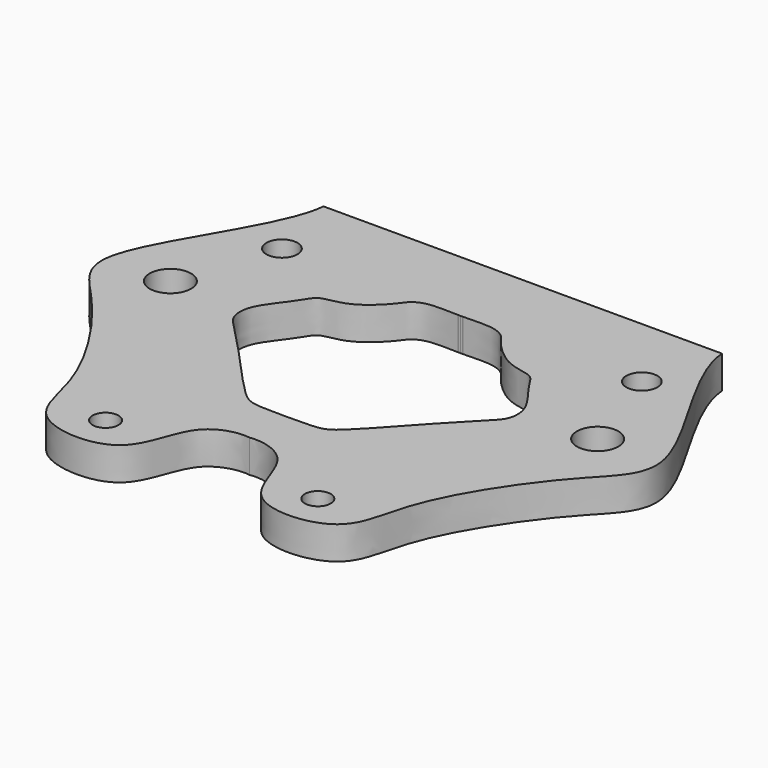
from build123d import *

# Parameters (mm, degrees)
F1_R     = 2.5
F1_R_2   = 4
F1_R_3   = 3
F2_DEPTH = 6.35


with BuildPart() as f2:
    # F1 (on Top) → F2 (new body)
    with BuildSketch(Plane.XY):
        with BuildLine():
            Line((0, 43.1096181273), (-38.4708940983, 43.1096181273))
            add(Edge.make_bspline(
                [(-38.4708940983, 43.1096181273), (-39.2133427516, 33.9005949369), (-59.8892548764, 9.0952637911), (-46.0173675583, -1.6874026228), (-31.2559828648, -23.675526799), (-31.0559444564, -38.9669124435), (-10.6108497143, -40.2396591076), (-9.979392721, -24.0203075199), (-2.0148781437, -22.454328045), (0, -22.8310581297)],
                knots=[0, 0, 0, 0, 0.2098097793, 0.3396923098, 0.5186124178, 0.6453813724, 0.7753975326, 0.9014531464, 1, 1, 1, 1], degree=3))
            add(Edge.make_bspline(
                [(38.4708940983, 43.1096181273), (39.2133427516, 33.9005949369), (59.8892548764, 9.0952637911), (46.0173675583, -1.6874026228), (31.2559828648, -23.675526799), (31.0559444564, -38.9669124435), (10.6108497143, -40.2396591076), (9.979392721, -24.0203075199), (2.0148781437, -22.454328045), (0, -22.8310581297)],
                knots=[0, 0, 0, 0, 0.2098097793, 0.3396923098, 0.5186124178, 0.6453813724, 0.7753975326, 0.9014531464, 1, 1, 1, 1], degree=3))
            Line((38.4708940983, 43.1096181273), (0, 43.1096181273))
        make_face()
        with Locations((-20.5, -31.9710049892)):
            Circle(F1_R, mode=Mode.SUBTRACT)
        with Locations((20.5, -31.9710049892)):
            Circle(F1_R, mode=Mode.SUBTRACT)
        with Locations((-41.25, 9.6289950108)):
            Circle(F1_R_2, mode=Mode.SUBTRACT)
        with BuildLine():
            add(Edge.make_bspline(
                [(6.4e-09, 33.0979972724), (-0.0882795025, 33.2592999344), (-0.3332425852, 32.9819845601), (-1.0451951422, 33.1579334113), (-2.2487974802, 33.1411417676), (-3.3407961239, 33.1859683537), (-4.2948911131, 33.1744516968), (-5.0282816557, 33.1539777391), (-5.6622169162, 33.1118427901), (-6.1870307796, 33.0570546815), (-6.5952289435, 33.0054743687), (-7.0102229618, 32.9395197968), (-7.5499388032, 32.838326809), (-8.2016195007, 32.6840216918), (-8.965130544, 32.4416980665), (-9.7061375721, 32.1444970333), (-10.4238483213, 31.7898805655), (-11.1127698203, 31.3737269113), (-11.6598301582, 30.9662942141), (-12.0817470008, 30.598875736), (-12.4703312416, 30.2379058719), (-12.8750626777, 29.8002006617), (-13.2396391484, 29.3421168897), (-13.5155937125, 28.9712158097), (-13.735521076, 28.6712182084), (-13.8987403031, 28.4560361242), (-14.0298406312, 28.290951545), (-14.1756556012, 28.1118526983), (-14.3896915822, 27.8601939958), (-14.7795104996, 27.4279747105), (-15.3291303008, 26.8644903549), (-15.9424077049, 26.3272137222), (-16.4429773739, 25.9420418037), (-16.801971962, 25.6874882614), (-17.1341630528, 25.4773498972), (-17.37987551, 25.3463509203), (-17.5430523692, 25.2693490183), (-17.6781905661, 25.2106760658), (-17.8236093268, 25.1536978218), (-18.0332337047, 25.0779102475), (-18.3188446939, 24.9882243484), (-18.7075777861, 24.886621506), (-19.1386357508, 24.7880197301), (-19.6151193446, 24.6873703807), (-20.1460597766, 24.5750792354), (-20.6395911181, 24.4610958033), (-21.0977457597, 24.3327353739), (-21.411617551, 24.2343461901), (-21.6930929181, 24.1340464324), (-21.9889609382, 24.021743024), (-22.5176696762, 23.8006035335), (-23.249083116, 23.4084143093), (-24.0282071216, 22.8091400188), (-24.6397517452, 22.1843671352), (-25.0089456992, 21.7155994015), (-25.2445576365, 21.3991672419), (-25.4468239327, 21.118243955), (-25.6765867676, 20.7815619377), (-25.9273267838, 20.3978180586), (-26.1692884992, 20.0212779518), (-26.4096317036, 19.6465202567), (-26.6491002111, 19.2777095768), (-26.892256865, 18.9117109471), (-27.1045042906, 18.6038372115), (-27.2793693031, 18.3585097171), (-27.469301205, 18.0960354455), (-27.7375832378, 17.7347273013), (-28.0888266147, 17.26832658), (-28.5996228639, 16.5838499027), (-29.1397322152, 15.8490576463), (-29.699857386, 14.9922780094), (-30.1130401748, 14.3173197631), (-30.5240660906, 13.5691851268), (-30.8386957399, 12.8985424575), (-31.0750085695, 12.3043128456), (-31.2932342334, 11.7071680746), (-31.5196927833, 10.946253681), (-31.7042454361, 10.0433989464), (-31.8655515261, 8.8147451825), (-31.8601694529, 7.6086455946), (-31.6593056893, 6.366232041), (-31.4359894469, 5.4549728547), (-31.106635517, 4.5339965806), (-30.6899056673, 3.6894509534), (-30.2355331699, 2.9506780353), (-29.6049890767, 2.0685235743), (-28.9902998629, 1.4027333345), (-28.3974197119, 0.7885262776), (-28.0400082398, 0.4317039018), (-27.7497866964, 0.1407617436), (-27.4697942529, -0.1396146952), (-27.0989589964, -0.5145500465), (-26.6302533589, -0.992645741), (-25.965257484, -1.6755292824), (-25.0908248246, -2.5826074879), (-23.9691358159, -3.760933765), (-22.8023252814, -4.999304995), (-21.5955699779, -6.2932368866), (-20.3800075182, -7.6084418076), (-19.1772293001, -8.9265236382), (-17.9844679131, -10.2441462938), (-16.8120013991, -11.5336879547), (-15.6819278108, -12.7600431118), (-14.5841560667, -13.9191433001), (-13.7046780858, -14.8039966228), (-12.992643826, -15.4780561372), (-12.4656636682, -15.956298516), (-11.9243054801, -16.4201466396), (-11.3368108249, -16.8796778914), (-10.6813988035, -17.3301215836), (-9.9493095336, -17.753190934), (-9.1604307911, -18.1191766165), (-8.336002452, -18.411648255), (-7.6371691134, -18.5856032503), (-7.082822246, -18.6932766525), (-6.5247041187, -18.7869800741), (-5.8723669202, -18.8622713081), (-4.8723500771, -18.9386684681), (-3.7069059188, -18.9694473122), (-2.4014581908, -18.9505592756), (-1.2388662832, -19.0048677159), (-0.5840056397, -18.8877085009), (-0.2703453363, -19.2772670602), (-0.0970635213, -18.0762262208), (0, -16.9243552215)],
                knots=[0, 0, 0, 0, 0.0051702697, 0.0129899519, 0.0233308075, 0.0332171653, 0.0422856594, 0.050270348, 0.0576947557, 0.0644473849, 0.0703803284, 0.0763755892, 0.0832518239, 0.0909150243, 0.0992761376, 0.1076263044, 0.1159846149, 0.1243720614, 0.1320736917, 0.1390027554, 0.1457692734, 0.1529915951, 0.1601592135, 0.1665205175, 0.1721900714, 0.1770036811, 0.1812398876, 0.1856463316, 0.190943484, 0.198034366, 0.2064081222, 0.2149071862, 0.222294832, 0.2284725985, 0.2343079591, 0.2392171416, 0.2431356105, 0.2466641987, 0.250318881, 0.2546837164, 0.2597965273, 0.2657131994, 0.2719289285, 0.2784508345, 0.2853270785, 0.292028944, 0.2984432584, 0.3037893765, 0.3087907869, 0.3139791756, 0.3209550274, 0.3295125685, 0.338841997, 0.347608715, 0.3547659055, 0.3605452011, 0.3659815705, 0.3719286804, 0.3782644982, 0.3845190291, 0.3907310961, 0.396933472, 0.403138406, 0.4088329684, 0.4139051518, 0.4191680846, 0.4253636634, 0.4325082206, 0.4411029256, 0.4501321675, 0.4595305326, 0.4678829373, 0.4764642599, 0.4845153812, 0.491916261, 0.4993214992, 0.5075610259, 0.5165524669, 0.526906816, 0.5372635678, 0.5476663614, 0.5567222588, 0.5658981731, 0.5749080835, 0.5836294315, 0.5932946496, 0.6023163718, 0.6108818408, 0.61749732, 0.6233725505, 0.6292127725, 0.635923059, 0.6435387824, 0.6525905435, 0.6630903437, 0.675010275, 0.6872282029, 0.6996333082, 0.7121232758, 0.7245878425, 0.7370299222, 0.7493404338, 0.7614338298, 0.7732336215, 0.7836894943, 0.7928454913, 0.8006749239, 0.8084946868, 0.8165494609, 0.8248658513, 0.8334367931, 0.8421668266, 0.8509192432, 0.8588204572, 0.8657899233, 0.8727126261, 0.8802409656, 0.8895415172, 0.8996893499, 0.9104543574, 0.9206204255, 0.9280336121, 0.932673258, 0.939906013, 0.939906013, 0.939906013, 0.939906013], degree=3))
            add(Edge.make_bspline(
                [(-6.4e-09, 33.0979972724), (0.0882795025, 33.2592999344), (0.3332425852, 32.9819845601), (1.0451951422, 33.1579334113), (2.2487974802, 33.1411417676), (3.3407961239, 33.1859683537), (4.2948911131, 33.1744516968), (5.0282816557, 33.1539777391), (5.6622169162, 33.1118427901), (6.1870307796, 33.0570546815), (6.5952289435, 33.0054743687), (7.0102229618, 32.9395197968), (7.5499388032, 32.838326809), (8.2016195007, 32.6840216918), (8.965130544, 32.4416980665), (9.7061375721, 32.1444970333), (10.4238483213, 31.7898805655), (11.1127698203, 31.3737269113), (11.6598301582, 30.9662942141), (12.0817470008, 30.598875736), (12.4703312416, 30.2379058719), (12.8750626777, 29.8002006617), (13.2396391484, 29.3421168897), (13.5155937125, 28.9712158097), (13.735521076, 28.6712182084), (13.8987403031, 28.4560361242), (14.0298406312, 28.290951545), (14.1756556012, 28.1118526983), (14.3896915822, 27.8601939958), (14.7795104996, 27.4279747105), (15.3291303008, 26.8644903549), (15.9424077049, 26.3272137222), (16.4429773739, 25.9420418037), (16.801971962, 25.6874882614), (17.1341630528, 25.4773498972), (17.37987551, 25.3463509203), (17.5430523692, 25.2693490183), (17.6781905661, 25.2106760658), (17.8236093268, 25.1536978218), (18.0332337047, 25.0779102475), (18.3188446939, 24.9882243484), (18.7075777861, 24.886621506), (19.1386357508, 24.7880197301), (19.6151193446, 24.6873703807), (20.1460597766, 24.5750792354), (20.6395911181, 24.4610958033), (21.0977457597, 24.3327353739), (21.411617551, 24.2343461901), (21.6930929181, 24.1340464324), (21.9889609382, 24.021743024), (22.5176696762, 23.8006035335), (23.249083116, 23.4084143093), (24.0282071216, 22.8091400188), (24.6397517452, 22.1843671352), (25.0089456992, 21.7155994015), (25.2445576365, 21.3991672419), (25.4468239327, 21.118243955), (25.6765867676, 20.7815619377), (25.9273267838, 20.3978180586), (26.1692884992, 20.0212779518), (26.4096317036, 19.6465202567), (26.6491002111, 19.2777095768), (26.892256865, 18.9117109471), (27.1045042906, 18.6038372115), (27.2793693031, 18.3585097171), (27.469301205, 18.0960354455), (27.7375832378, 17.7347273013), (28.0888266147, 17.26832658), (28.5996228639, 16.5838499027), (29.1397322152, 15.8490576463), (29.699857386, 14.9922780094), (30.1130401748, 14.3173197631), (30.5240660906, 13.5691851268), (30.8386957399, 12.8985424575), (31.0750085695, 12.3043128456), (31.2932342334, 11.7071680746), (31.5196927833, 10.946253681), (31.7042454361, 10.0433989464), (31.8655515261, 8.8147451825), (31.8601694529, 7.6086455946), (31.6593056893, 6.366232041), (31.4359894469, 5.4549728547), (31.106635517, 4.5339965806), (30.6899056673, 3.6894509534), (30.2355331699, 2.9506780353), (29.6049890767, 2.0685235743), (28.9902998629, 1.4027333345), (28.3974197119, 0.7885262776), (28.0400082398, 0.4317039018), (27.7497866964, 0.1407617436), (27.4697942529, -0.1396146952), (27.0989589964, -0.5145500465), (26.6302533589, -0.992645741), (25.965257484, -1.6755292824), (25.0908248246, -2.5826074879), (23.9691358159, -3.760933765), (22.8023252814, -4.999304995), (21.5955699779, -6.2932368866), (20.3800075182, -7.6084418076), (19.1772293001, -8.9265236382), (17.9844679131, -10.2441462938), (16.8120013991, -11.5336879547), (15.6819278108, -12.7600431118), (14.5841560667, -13.9191433001), (13.7046780858, -14.8039966228), (12.992643826, -15.4780561372), (12.4656636682, -15.956298516), (11.9243054801, -16.4201466396), (11.3368108249, -16.8796778914), (10.6813988035, -17.3301215836), (9.9493095336, -17.753190934), (9.1604307911, -18.1191766165), (8.336002452, -18.411648255), (7.6371691134, -18.5856032503), (7.082822246, -18.6932766525), (6.5247041187, -18.7869800741), (5.8723669202, -18.8622713081), (4.8723500771, -18.9386684681), (3.7069059188, -18.9694473122), (2.4014581908, -18.9505592756), (1.2388662832, -19.0048677159), (0.5840056397, -18.8877085009), (0.2703453363, -19.2772670602), (0.0970635213, -18.0762262208), (0, -16.9243552215)],
                knots=[0, 0, 0, 0, 0.0051702697, 0.0129899519, 0.0233308075, 0.0332171653, 0.0422856594, 0.050270348, 0.0576947557, 0.0644473849, 0.0703803284, 0.0763755892, 0.0832518239, 0.0909150243, 0.0992761376, 0.1076263044, 0.1159846149, 0.1243720614, 0.1320736917, 0.1390027554, 0.1457692734, 0.1529915951, 0.1601592135, 0.1665205175, 0.1721900714, 0.1770036811, 0.1812398876, 0.1856463316, 0.190943484, 0.198034366, 0.2064081222, 0.2149071862, 0.222294832, 0.2284725985, 0.2343079591, 0.2392171416, 0.2431356105, 0.2466641987, 0.250318881, 0.2546837164, 0.2597965273, 0.2657131994, 0.2719289285, 0.2784508345, 0.2853270785, 0.292028944, 0.2984432584, 0.3037893765, 0.3087907869, 0.3139791756, 0.3209550274, 0.3295125685, 0.338841997, 0.347608715, 0.3547659055, 0.3605452011, 0.3659815705, 0.3719286804, 0.3782644982, 0.3845190291, 0.3907310961, 0.396933472, 0.403138406, 0.4088329684, 0.4139051518, 0.4191680846, 0.4253636634, 0.4325082206, 0.4411029256, 0.4501321675, 0.4595305326, 0.4678829373, 0.4764642599, 0.4845153812, 0.491916261, 0.4993214992, 0.5075610259, 0.5165524669, 0.526906816, 0.5372635678, 0.5476663614, 0.5567222588, 0.5658981731, 0.5749080835, 0.5836294315, 0.5932946496, 0.6023163718, 0.6108818408, 0.61749732, 0.6233725505, 0.6292127725, 0.635923059, 0.6435387824, 0.6525905435, 0.6630903437, 0.675010275, 0.6872282029, 0.6996333082, 0.7121232758, 0.7245878425, 0.7370299222, 0.7493404338, 0.7614338298, 0.7732336215, 0.7836894943, 0.7928454913, 0.8006749239, 0.8084946868, 0.8165494609, 0.8248658513, 0.8334367931, 0.8421668266, 0.8509192432, 0.8588204572, 0.8657899233, 0.8727126261, 0.8802409656, 0.8895415172, 0.8996893499, 0.9104543574, 0.9206204255, 0.9280336121, 0.932673258, 0.939906013, 0.939906013, 0.939906013, 0.939906013], degree=3))
        make_face(mode=Mode.SUBTRACT)
        with Locations((-34.75, 28.4289950108)):
            Circle(F1_R_3, mode=Mode.SUBTRACT)
        with Locations((41.25, 9.6289950108)):
            Circle(F1_R_2, mode=Mode.SUBTRACT)
        with Locations((34.75, 28.4289950108)):
            Circle(F1_R_3, mode=Mode.SUBTRACT)
        with BuildLine():
            add(Edge.make_bspline(
                [(0, 28.0979972724), (-0.1387467144, 28.0979972726), (-0.2796740198, 28.0990707052), (-0.4223904323, 28.1009624133)],
                knots=[0, 0, 0, 0, 0.0057440238, 0.0057440238, 0.0057440238, 0.0057440238], degree=3))
            add(Edge.make_bspline(
                [(0, 28.0979972724), (0.1387467144, 28.0979972726), (0.2796740198, 28.0990707052), (0.4223904323, 28.1009624133)],
                knots=[0, 0, 0, 0, 0.0057440238, 0.0057440238, 0.0057440238, 0.0057440238], degree=3))
            add(Edge.make_bspline(
                [(0.4223904326, 28.1009624134), (0.3121432838, 30.0279508852), (0.1720583206, 31.287921758), (4.5e-09, 31.5979968295)],
                knots=[0.9893651803, 0.9893651803, 0.9893651803, 0.9893651803, 1, 1, 1, 1], degree=3))
            add(Edge.make_bspline(
                [(-0.4223904326, 28.1009624134), (-0.3121432838, 30.0279508852), (-0.1720583206, 31.287921758), (-4.5e-09, 31.5979968295)],
                knots=[0.9893651803, 0.9893651803, 0.9893651803, 0.9893651803, 1, 1, 1, 1], degree=3))
        make_face()
        with BuildLine():
            add(Edge.make_bspline(
                [(-0.4223904323, 28.1009624133), (-0.4251966179, 28.1009996094), (-0.4280034951, 28.1010371218), (-0.4308110611, 28.1010749486)],
                knots=[0.0057440238, 0.0057440238, 0.0057440238, 0.0057440238, 0.0058569667, 0.0058569667, 0.0058569667, 0.0058569667], degree=3))
            add(Edge.make_bspline(
                [(-0.4223904326, 28.1009624134), (-0.3121432838, 30.0279508852), (-0.1720583206, 31.287921758), (-4.5e-09, 31.5979968295)],
                knots=[0.9893651803, 0.9893651803, 0.9893651803, 0.9893651803, 1, 1, 1, 1], degree=3))
            add(Edge.make_bspline(
                [(4.5e-09, 31.5979968295), (-0.0176621206, 31.6298266464), (-0.0356611626, 31.6516470058), (-0.0540950125, 31.6657370126)],
                knots=[0, 0, 0, 0, 0.0010916852, 0.0010916852, 0.0010916852, 0.0010916852], degree=3))
            add(Edge.make_bspline(
                [(-0.4308110613, 28.1010749486), (-0.3313602574, 29.9299947273), (-0.2063777094, 31.1929840288), (-0.0540950125, 31.6657370126)],
                knots=[0.9891940627, 0.9891940627, 0.9891940627, 0.9891940627, 0.9988768785, 0.9988768785, 0.9988768785, 0.9988768785], degree=3))
        make_face()
        with BuildLine():
            add(Edge.make_bspline(
                [(0.4223904326, 28.1009624134), (0.3121432838, 30.0279508852), (0.1720583206, 31.287921758), (4.5e-09, 31.5979968295)],
                knots=[0.9893651803, 0.9893651803, 0.9893651803, 0.9893651803, 1, 1, 1, 1], degree=3))
            add(Edge.make_bspline(
                [(0.4223904323, 28.1009624133), (0.4251966179, 28.1009996094), (0.4280034951, 28.1010371218), (0.4308110611, 28.1010749486)],
                knots=[0.0057440238, 0.0057440238, 0.0057440238, 0.0057440238, 0.0058569667, 0.0058569667, 0.0058569667, 0.0058569667], degree=3))
            add(Edge.make_bspline(
                [(0.4308110613, 28.1010749486), (0.3313602574, 29.9299947273), (0.2063777094, 31.1929840288), (0.0540950125, 31.6657370126)],
                knots=[0.9891940627, 0.9891940627, 0.9891940627, 0.9891940627, 0.9988768785, 0.9988768785, 0.9988768785, 0.9988768785], degree=3))
            add(Edge.make_bspline(
                [(-4.5e-09, 31.5979968295), (0.0176621206, 31.6298266464), (0.0356611626, 31.6516470058), (0.0540950125, 31.6657370126)],
                knots=[0, 0, 0, 0, 0.0010916852, 0.0010916852, 0.0010916852, 0.0010916852], degree=3))
        make_face()
        with BuildLine():
            add(Edge.make_bspline(
                [(-0.4308110611, 28.1010749486), (-0.4442409472, 28.1012558917), (-0.4576865926, 28.1014440293), (-0.4711476714, 28.1016391491)],
                knots=[0.0058569667, 0.0058569667, 0.0058569667, 0.0058569667, 0.0063972245, 0.0063972245, 0.0063972245, 0.0063972245], degree=3))
            add(Edge.make_bspline(
                [(-0.4308110613, 28.1010749486), (-0.3313602574, 29.9299947273), (-0.2063777094, 31.1929840288), (-0.0540950125, 31.6657370126)],
                knots=[0.9891940627, 0.9891940627, 0.9891940627, 0.9891940627, 0.9988768785, 0.9988768785, 0.9988768785, 0.9988768785], degree=3))
            add(Edge.make_bspline(
                [(-0.0540950125, 31.6657370126), (-0.1161284756, 31.7131526052), (-0.1830859324, 31.6730256355), (-0.2586979361, 31.632210997)],
                knots=[0.0010916852, 0.0010916852, 0.0010916852, 0.0010916852, 0.0047654166, 0.0047654166, 0.0047654166, 0.0047654166], degree=3))
            add(Edge.make_bspline(
                [(-0.4711476716, 28.1016391491), (-0.412883937, 29.564117131), (-0.3423220818, 30.7663792887), (-0.2586979381, 31.6322109988)],
                knots=[0.9879914698, 0.9879914698, 0.9879914698, 0.9879914698, 0.9943054354, 0.9943054354, 0.9943054354, 0.9943054354], degree=3))
        make_face()
        with BuildLine():
            add(Edge.make_bspline(
                [(4.5e-09, 31.5979968295), (-0.0176621206, 31.6298266464), (-0.0356611626, 31.6516470058), (-0.0540950125, 31.6657370126)],
                knots=[0, 0, 0, 0, 0.0010916852, 0.0010916852, 0.0010916852, 0.0010916852], degree=3))
            add(Edge.make_bspline(
                [(-4.5e-09, 31.5979968295), (0.0176621206, 31.6298266464), (0.0356611626, 31.6516470058), (0.0540950125, 31.6657370126)],
                knots=[0, 0, 0, 0, 0.0010916852, 0.0010916852, 0.0010916852, 0.0010916852], degree=3))
            add(Edge.make_bspline(
                [(0.0540950125, 31.6657370126), (0.0364315583, 31.7205722031), (0.0184008089, 31.7647755852), (4.8e-09, 31.7979971204)],
                knots=[0.9988768785, 0.9988768785, 0.9988768785, 0.9988768785, 1, 1, 1, 1], degree=3))
            add(Edge.make_bspline(
                [(-0.0540950125, 31.6657370126), (-0.0364315583, 31.7205722031), (-0.0184008089, 31.7647755852), (-4.8e-09, 31.7979971204)],
                knots=[0.9988768785, 0.9988768785, 0.9988768785, 0.9988768785, 1, 1, 1, 1], degree=3))
        make_face()
        with BuildLine():
            add(Edge.make_bspline(
                [(0.4308110613, 28.1010749486), (0.3313602574, 29.9299947273), (0.2063777094, 31.1929840288), (0.0540950125, 31.6657370126)],
                knots=[0.9891940627, 0.9891940627, 0.9891940627, 0.9891940627, 0.9988768785, 0.9988768785, 0.9988768785, 0.9988768785], degree=3))
            add(Edge.make_bspline(
                [(0.4308110611, 28.1010749486), (0.4442409472, 28.1012558917), (0.4576865926, 28.1014440293), (0.4711476714, 28.1016391491)],
                knots=[0.0058569667, 0.0058569667, 0.0058569667, 0.0058569667, 0.0063972245, 0.0063972245, 0.0063972245, 0.0063972245], degree=3))
            add(Edge.make_bspline(
                [(0.4711476716, 28.1016391491), (0.412883937, 29.564117131), (0.3423220818, 30.7663792887), (0.2586979381, 31.6322109988)],
                knots=[0.9879914698, 0.9879914698, 0.9879914698, 0.9879914698, 0.9943054354, 0.9943054354, 0.9943054354, 0.9943054354], degree=3))
            add(Edge.make_bspline(
                [(0.0540950125, 31.6657370126), (0.1161284756, 31.7131526052), (0.1830859324, 31.6730256355), (0.2586979361, 31.632210997)],
                knots=[0.0010916852, 0.0010916852, 0.0010916852, 0.0010916852, 0.0047654166, 0.0047654166, 0.0047654166, 0.0047654166], degree=3))
        make_face()
        with BuildLine():
            add(Edge.make_bspline(
                [(-0.4711476714, 28.1016391491), (-2.2737445474, 28.1277679813), (-5.9467320288, 28.3950878552), (-8.8491155492, 27.1034023416), (-10.0259101427, 25.0140002486), (-14.9376610538, 20.0597479872), (-20.0675972196, 19.7490636744), (-21.3356691631, 18.4137052745), (-23.1244711188, 15.3160147238), (-26.8933353014, 10.9021150336), (-26.9715954823, 6.3448369246), (-23.7856739849, 3.3333814129), (-16.1507032946, -4.7150900938), (-9.3910531365, -12.3914442147), (-6.2965356963, -14.1615775488), (-2.028846852, -13.9105881243), (-0.2149320674, -14.0026022136)],
                knots=[0.0063972245, 0.0063972245, 0.0063972245, 0.0063972245, 0.0787441042, 0.1341912789, 0.1833675971, 0.2678740922, 0.3391372862, 0.3798203274, 0.4402520286, 0.5186622798, 0.5827313378, 0.6475508766, 0.7572933281, 0.8606783417, 0.9205896248, 0.9969440739, 0.9969440739, 0.9969440739, 0.9969440739], degree=3))
            add(Edge.make_bspline(
                [(-0.4711476716, 28.1016391491), (-0.412883937, 29.564117131), (-0.3423220818, 30.7663792887), (-0.2586979381, 31.6322109988)],
                knots=[0.9879914698, 0.9879914698, 0.9879914698, 0.9879914698, 0.9943054354, 0.9943054354, 0.9943054354, 0.9943054354], degree=3))
            add(Edge.make_bspline(
                [(-0.2586979361, 31.632210997), (-0.2811109979, 31.62011264), (-0.48982217, 31.5106051029), (-1.0895646814, 31.6595083238), (-2.293190841, 31.6418206496), (-3.3562668496, 31.6856007465), (-4.2737453965, 31.67424907), (-4.9599987337, 31.6550043344), (-5.6624202696, 31.6100096214), (-6.2551620508, 31.5428362762), (-6.7440384233, 31.4625861764), (-7.2217019082, 31.3733915513), (-7.7977126994, 31.2370246306), (-8.4570994188, 31.0273643211), (-9.0924157023, 30.7724522644), (-9.7004163725, 30.4717390667), (-10.2775746086, 30.1229569854), (-10.7314856216, 29.7843851404), (-11.07705262, 29.483830589), (-11.4031227604, 29.180030146), (-11.7389175593, 28.8176843169), (-12.1705716058, 28.2866319513), (-12.4517417233, 27.8755796021), (-12.7100538632, 27.5414755752), (-12.8589134896, 27.3530505792), (-13.0279975796, 27.1455985276), (-13.2652191304, 26.8668191468), (-13.6951328817, 26.39014406), (-14.2972374927, 25.77312261), (-14.9768011451, 25.1766735407), (-15.546068745, 24.7385000119), (-15.9654399821, 24.4406999124), (-16.3703740232, 24.1842851542), (-16.6899915717, 24.0125469361), (-16.9248982457, 23.9019278076), (-17.1706745723, 23.7940149855), (-17.4923276529, 23.6726496965), (-17.9068507984, 23.5449966972), (-18.3471807293, 23.4301216271), (-18.8151507706, 23.3232558018), (-19.3057184629, 23.2194271425), (-19.8229103827, 23.1109326979), (-20.3811483532, 22.9795378707), (-20.9935654901, 22.8122045825), (-21.7177355779, 22.5364789997), (-22.4100407549, 22.1507838461), (-23.0361204628, 21.6716248788), (-23.5276113839, 21.1708104525), (-23.8971318236, 20.708298236), (-24.1704471522, 20.3270631967), (-24.4264497266, 19.9527854366), (-24.6680879233, 19.5825707251), (-24.9077461724, 19.2098485397), (-25.149600277, 18.8326575903), (-25.3956720513, 18.4536327541), (-25.6497347593, 18.0712045104), (-25.8738674034, 17.7459705934), (-26.061187968, 17.4831883682), (-26.2610223715, 17.207072351), (-26.5353510115, 16.8377346829), (-26.8915583546, 16.3645804651), (-27.3931904722, 15.69268541), (-28.0507916991, 14.7981440732), (-28.6974456181, 13.7989288704), (-29.1821073795, 12.8928435862), (-29.5276047091, 12.1700252399), (-29.8293188325, 11.3853171978), (-30.056885282, 10.5977144761), (-30.2205460495, 9.7993694153), (-30.3604290549, 8.7366155902), (-30.3691080408, 7.4319011073), (-30.1039286323, 6.1372259563), (-29.718156431, 5.1243900199), (-29.2706739647, 4.1643758559), (-28.5963735283, 3.1817139527), (-27.7500963594, 2.2562677567), (-27.1289608133, 1.6436363419), (-26.6938557903, 1.2058903509), (-26.4090034788, 0.9209958915), (-26.0287038345, 0.5364390351), (-25.5569992978, 0.0552638951), (-24.8892326887, -0.6303862255), (-23.996196306, -1.5569825563), (-22.8697462523, -2.7402053105), (-21.2903446309, -4.4148527529), (-19.697956161, -6.1279949576), (-18.0758295781, -7.9082627585), (-16.8873226516, -9.2210030353), (-15.7024889399, -10.5242578775), (-14.587128869, -11.7344808165), (-13.5067184582, -12.8752761351), (-12.6520373951, -13.7347388957), (-11.9712475951, -14.3791710664), (-11.4740441217, -14.8302235974), (-10.9772465026, -15.2557323667), (-10.4459377598, -15.6706805078), (-9.8764036057, -16.0595003762), (-9.0486631203, -16.5547962769), (-8.130971648, -16.9271998589), (-7.1677419832, -17.1595223584), (-6.2037815158, -17.3428754283), (-5.0461419832, -17.4335313108), (-3.6914874736, -17.4708240644), (-2.40894479, -17.4498798718), (-1.2178733399, -17.5072875124), (-0.5250476476, -17.3793070658), (-0.2301440546, -17.7392396034), (-0.0854383204, -17.0932504356), (-0.022740778, -16.6448680684)],
                knots=[0.0047654166, 0.0047654166, 0.0047654166, 0.0047654166, 0.0058543914, 0.0145732225, 0.0259032088, 0.036593093, 0.0462936016, 0.0547675915, 0.0633149064, 0.0712207813, 0.078357526, 0.0854317625, 0.0932852015, 0.1018094643, 0.1102764707, 0.1187048207, 0.1271151154, 0.1347949679, 0.1416755583, 0.1484080397, 0.1556379886, 0.1640917075, 0.1714364231, 0.1779706251, 0.1829478323, 0.1881065095, 0.1942308174, 0.2023817771, 0.2119778206, 0.2217793194, 0.2304119209, 0.2377289731, 0.2447900151, 0.2509239331, 0.2560742438, 0.2613068859, 0.267290227, 0.274033586, 0.2809482959, 0.2880205772, 0.2952525706, 0.3026753082, 0.310383748, 0.318528183, 0.3275129007, 0.3366435735, 0.3457156065, 0.35429369, 0.362122518, 0.3691011319, 0.3759507636, 0.3827456991, 0.389543753, 0.3963765959, 0.4032643181, 0.4102126957, 0.4166284086, 0.4223827936, 0.4282990162, 0.4351763966, 0.4430126393, 0.4523486291, 0.4631825841, 0.4744255416, 0.4847532187, 0.4938732907, 0.5032020143, 0.5124219402, 0.5215953553, 0.5321320891, 0.5438734425, 0.5556152154, 0.5662155594, 0.5766466321, 0.5878483778, 0.5993434945, 0.6089416809, 0.6168131511, 0.6232490205, 0.6306425979, 0.6390223672, 0.6489757836, 0.6605124332, 0.6736024633, 0.6890904354, 0.7049332948, 0.7207377382, 0.7343702018, 0.747830846, 0.7610182512, 0.7738355481, 0.7851237427, 0.7949292175, 0.8032552953, 0.8114774778, 0.8198088786, 0.828296253, 0.8383002109, 0.8485261793, 0.8586495499, 0.8687303417, 0.8797322251, 0.891647559, 0.9033576768, 0.9145833958, 0.9229774502, 0.9284013715, 0.9329627681, 0.9329627681, 0.9329627681, 0.9329627681], degree=3))
            add(Edge.make_bspline(
                [(-0.022740778, -16.6448680684), (-0.0475480751, -16.3293973516), (-0.0717783107, -15.9863087841), (-0.0954114894, -15.6175966251)],
                knots=[0.9404747926, 0.9404747926, 0.9404747926, 0.9404747926, 0.9423492834, 0.9423492834, 0.9423492834, 0.9423492834], degree=3))
            add(Edge.make_bspline(
                [(-0.0954114894, -15.6175966251), (-0.1176240622, -15.3614741867), (-0.1393224076, -15.0848063487), (-0.1604963584, -14.78888273)],
                knots=[0.9371288764, 0.9371288764, 0.9371288764, 0.9371288764, 0.9388635135, 0.9388635135, 0.9388635135, 0.9388635135], degree=3))
            add(Edge.make_bspline(
                [(-0.1604963584, -14.78888273), (-0.1790437456, -14.5410652517), (-0.19719108, -14.2786937741), (-0.2149320658, -14.0026022134)],
                knots=[0.937675382, 0.937675382, 0.937675382, 0.937675382, 0.9392002693, 0.9392002693, 0.9392002693, 0.9392002693], degree=3))
        make_face()
        with BuildLine():
            add(Edge.make_bspline(
                [(-0.0540950125, 31.6657370126), (-0.1161284756, 31.7131526052), (-0.1830859324, 31.6730256355), (-0.2586979361, 31.632210997)],
                knots=[0.0010916852, 0.0010916852, 0.0010916852, 0.0010916852, 0.0047654166, 0.0047654166, 0.0047654166, 0.0047654166], degree=3))
            add(Edge.make_bspline(
                [(-0.0540950125, 31.6657370126), (-0.0364315583, 31.7205722031), (-0.0184008089, 31.7647755852), (-4.8e-09, 31.7979971204)],
                knots=[0.9988768785, 0.9988768785, 0.9988768785, 0.9988768785, 1, 1, 1, 1], degree=3))
            add(Edge.make_bspline(
                [(4.8e-09, 31.7979971204), (-0.0713753065, 31.9268609133), (-0.1483184797, 31.890491318), (-0.2374485852, 31.8422829657)],
                knots=[0, 0, 0, 0, 0.0043565024, 0.0043565024, 0.0043565024, 0.0043565024], degree=3))
            add(Edge.make_bspline(
                [(-0.2586979381, 31.6322109988), (-0.2517062776, 31.7046015921), (-0.2446233074, 31.7746404277), (-0.237448581, 31.842282962)],
                knots=[0.9943054354, 0.9943054354, 0.9943054354, 0.9943054354, 0.9948333344, 0.9948333344, 0.9948333344, 0.9948333344], degree=3))
        make_face()
        with BuildLine():
            add(Edge.make_bspline(
                [(-0.1035831912, -15.4887081413), (-0.1323162279, -15.0305798825), (-0.1601528468, -14.5344736488), (-0.1870564751, -14.0040370355)],
                knots=[0.942565966, 0.942565966, 0.942565966, 0.942565966, 0.9448583727, 0.9448583727, 0.9448583727, 0.9448583727], degree=3))
            add(Edge.make_bspline(
                [(-0.2127663331, -14.0027121989), (-0.2041833857, -14.0031485718), (-0.1956133851, -14.0035901619), (-0.1870564758, -14.0040370356)],
                knots=[0.9969744657, 0.9969744657, 0.9969744657, 0.9969744657, 0.9973358456, 0.9973358456, 0.9973358456, 0.9973358456], degree=3))
            add(Edge.make_bspline(
                [(-0.1604963584, -14.78888273), (-0.1782921085, -14.5401722825), (-0.195717445, -14.2778602371), (-0.2127663318, -14.0027121987)],
                knots=[0.9388635135, 0.9388635135, 0.9388635135, 0.9388635135, 0.9403213976, 0.9403213976, 0.9403213976, 0.9403213976], degree=3))
            add(Edge.make_bspline(
                [(-0.1035831912, -15.4887081413), (-0.1229511505, -15.2705838915), (-0.1419243131, -15.0370296722), (-0.1604963584, -14.78888273)],
                knots=[0.9361484674, 0.9361484674, 0.9361484674, 0.9361484674, 0.937675382, 0.937675382, 0.937675382, 0.937675382], degree=3))
        make_face()
        with BuildLine():
            add(Edge.make_bspline(
                [(-0.1870564758, -14.0040370356), (-0.1239734856, -14.0073314645), (-0.0616020002, -14.0109130549), (0, -14.0148084611)],
                knots=[0.9973358456, 0.9973358456, 0.9973358456, 0.9973358456, 1, 1, 1, 1], degree=3))
            add(Edge.make_bspline(
                [(-0.1035831912, -15.4887081413), (-0.1323162279, -15.0305798825), (-0.1601528468, -14.5344736488), (-0.1870564751, -14.0040370355)],
                knots=[0.942565966, 0.942565966, 0.942565966, 0.942565966, 0.9448583727, 0.9448583727, 0.9448583727, 0.9448583727], degree=3))
            add(Edge.make_bspline(
                [(0, -16.4743809385), (-0.0356779315, -16.1944730949), (-0.0702164347, -15.8644885007), (-0.1035831912, -15.4887081413)],
                knots=[0.9335179276, 0.9335179276, 0.9335179276, 0.9335179276, 0.9361484674, 0.9361484674, 0.9361484674, 0.9361484674], degree=3))
            add(Edge.make_bspline(
                [(0, -16.4743809385), (0.0356779315, -16.1944730949), (0.0702164347, -15.8644885007), (0.1035831912, -15.4887081413)],
                knots=[0.9335179276, 0.9335179276, 0.9335179276, 0.9335179276, 0.9361484674, 0.9361484674, 0.9361484674, 0.9361484674], degree=3))
            add(Edge.make_bspline(
                [(0.1035831912, -15.4887081413), (0.1323162279, -15.0305798825), (0.1601528468, -14.5344736488), (0.1870564751, -14.0040370355)],
                knots=[0.942565966, 0.942565966, 0.942565966, 0.942565966, 0.9448583727, 0.9448583727, 0.9448583727, 0.9448583727], degree=3))
            add(Edge.make_bspline(
                [(0.1870564758, -14.0040370356), (0.1239734856, -14.0073314645), (0.0616020002, -14.0109130549), (0, -14.0148084611)],
                knots=[0.9973358456, 0.9973358456, 0.9973358456, 0.9973358456, 1, 1, 1, 1], degree=3))
        make_face()
        with BuildLine():
            add(Edge.make_bspline(
                [(0.0540950125, 31.6657370126), (0.0364315583, 31.7205722031), (0.0184008089, 31.7647755852), (4.8e-09, 31.7979971204)],
                knots=[0.9988768785, 0.9988768785, 0.9988768785, 0.9988768785, 1, 1, 1, 1], degree=3))
            add(Edge.make_bspline(
                [(0.0540950125, 31.6657370126), (0.1161284756, 31.7131526052), (0.1830859324, 31.6730256355), (0.2586979361, 31.632210997)],
                knots=[0.0010916852, 0.0010916852, 0.0010916852, 0.0010916852, 0.0047654166, 0.0047654166, 0.0047654166, 0.0047654166], degree=3))
            add(Edge.make_bspline(
                [(0.2586979381, 31.6322109988), (0.2517062776, 31.7046015921), (0.2446233074, 31.7746404277), (0.237448581, 31.842282962)],
                knots=[0.9943054354, 0.9943054354, 0.9943054354, 0.9943054354, 0.9948333344, 0.9948333344, 0.9948333344, 0.9948333344], degree=3))
            add(Edge.make_bspline(
                [(-4.8e-09, 31.7979971204), (0.0713753065, 31.9268609132), (0.1483184797, 31.890491318), (0.2374485852, 31.8422829657)],
                knots=[0, 0, 0, 0, 0.0043565024, 0.0043565024, 0.0043565024, 0.0043565024], degree=3))
        make_face()
        with BuildLine():
            add(Edge.make_bspline(
                [(0.4711476716, 28.1016391491), (0.412883937, 29.564117131), (0.3423220818, 30.7663792887), (0.2586979381, 31.6322109988)],
                knots=[0.9879914698, 0.9879914698, 0.9879914698, 0.9879914698, 0.9943054354, 0.9943054354, 0.9943054354, 0.9943054354], degree=3))
            add(Edge.make_bspline(
                [(0.4711476714, 28.1016391491), (2.2737445474, 28.1277679813), (5.9467320288, 28.3950878552), (8.8491155492, 27.1034023416), (10.0259101427, 25.0140002486), (14.9376610538, 20.0597479872), (20.0675972196, 19.7490636744), (21.3356691631, 18.4137052745), (23.1244711188, 15.3160147238), (26.8933353014, 10.9021150336), (26.9715954823, 6.3448369246), (23.7856739849, 3.3333814129), (16.1507032946, -4.7150900938), (9.3910531365, -12.3914442147), (6.2965356963, -14.1615775488), (2.028846852, -13.9105881243), (0.2149320674, -14.0026022136)],
                knots=[0.0063972245, 0.0063972245, 0.0063972245, 0.0063972245, 0.0787441042, 0.1341912789, 0.1833675971, 0.2678740922, 0.3391372862, 0.3798203274, 0.4402520286, 0.5186622798, 0.5827313378, 0.6475508766, 0.7572933281, 0.8606783417, 0.9205896248, 0.9969440739, 0.9969440739, 0.9969440739, 0.9969440739], degree=3))
            add(Edge.make_bspline(
                [(0.1604963584, -14.78888273), (0.1790437456, -14.5410652517), (0.19719108, -14.2786937741), (0.2149320658, -14.0026022134)],
                knots=[0.937675382, 0.937675382, 0.937675382, 0.937675382, 0.9392002693, 0.9392002693, 0.9392002693, 0.9392002693], degree=3))
            add(Edge.make_bspline(
                [(0.0954114894, -15.6175966251), (0.1176240622, -15.3614741867), (0.1393224076, -15.0848063487), (0.1604963584, -14.78888273)],
                knots=[0.9371288764, 0.9371288764, 0.9371288764, 0.9371288764, 0.9388635135, 0.9388635135, 0.9388635135, 0.9388635135], degree=3))
            add(Edge.make_bspline(
                [(0.022740778, -16.6448680684), (0.0475480751, -16.3293973516), (0.0717783107, -15.9863087841), (0.0954114894, -15.6175966251)],
                knots=[0.9404747926, 0.9404747926, 0.9404747926, 0.9404747926, 0.9423492834, 0.9423492834, 0.9423492834, 0.9423492834], degree=3))
            add(Edge.make_bspline(
                [(0.2586979361, 31.632210997), (0.2811109979, 31.62011264), (0.48982217, 31.5106051029), (1.0895646814, 31.6595083238), (2.293190841, 31.6418206496), (3.3562668496, 31.6856007465), (4.2737453965, 31.67424907), (4.9599987337, 31.6550043344), (5.6624202696, 31.6100096214), (6.2551620508, 31.5428362762), (6.7440384233, 31.4625861764), (7.2217019082, 31.3733915513), (7.7977126994, 31.2370246306), (8.4570994188, 31.0273643211), (9.0924157023, 30.7724522644), (9.7004163725, 30.4717390667), (10.2775746086, 30.1229569854), (10.7314856216, 29.7843851404), (11.07705262, 29.483830589), (11.4031227604, 29.180030146), (11.7389175593, 28.8176843169), (12.1705716058, 28.2866319513), (12.4517417233, 27.8755796021), (12.7100538632, 27.5414755752), (12.8589134896, 27.3530505792), (13.0279975796, 27.1455985276), (13.2652191304, 26.8668191468), (13.6951328817, 26.39014406), (14.2972374927, 25.77312261), (14.9768011451, 25.1766735407), (15.546068745, 24.7385000119), (15.9654399821, 24.4406999124), (16.3703740232, 24.1842851542), (16.6899915717, 24.0125469361), (16.9248982457, 23.9019278076), (17.1706745723, 23.7940149855), (17.4923276529, 23.6726496965), (17.9068507984, 23.5449966972), (18.3471807293, 23.4301216271), (18.8151507706, 23.3232558018), (19.3057184629, 23.2194271425), (19.8229103827, 23.1109326979), (20.3811483532, 22.9795378707), (20.9935654901, 22.8122045825), (21.7177355779, 22.5364789997), (22.4100407549, 22.1507838461), (23.0361204628, 21.6716248788), (23.5276113839, 21.1708104525), (23.8971318236, 20.708298236), (24.1704471522, 20.3270631967), (24.4264497266, 19.9527854366), (24.6680879233, 19.5825707251), (24.9077461724, 19.2098485397), (25.149600277, 18.8326575903), (25.3956720513, 18.4536327541), (25.6497347593, 18.0712045104), (25.8738674034, 17.7459705934), (26.061187968, 17.4831883682), (26.2610223715, 17.207072351), (26.5353510115, 16.8377346829), (26.8915583546, 16.3645804651), (27.3931904722, 15.69268541), (28.0507916991, 14.7981440732), (28.6974456181, 13.7989288704), (29.1821073795, 12.8928435862), (29.5276047091, 12.1700252399), (29.8293188325, 11.3853171978), (30.056885282, 10.5977144761), (30.2205460495, 9.7993694153), (30.3604290549, 8.7366155902), (30.3691080408, 7.4319011073), (30.1039286323, 6.1372259563), (29.718156431, 5.1243900199), (29.2706739647, 4.1643758559), (28.5963735283, 3.1817139527), (27.7500963594, 2.2562677567), (27.1289608133, 1.6436363419), (26.6938557903, 1.2058903509), (26.4090034788, 0.9209958915), (26.0287038345, 0.5364390351), (25.5569992978, 0.0552638951), (24.8892326887, -0.6303862255), (23.996196306, -1.5569825563), (22.8697462523, -2.7402053105), (21.2903446309, -4.4148527529), (19.697956161, -6.1279949576), (18.0758295781, -7.9082627585), (16.8873226516, -9.2210030353), (15.7024889399, -10.5242578775), (14.587128869, -11.7344808165), (13.5067184582, -12.8752761351), (12.6520373951, -13.7347388957), (11.9712475951, -14.3791710664), (11.4740441217, -14.8302235974), (10.9772465026, -15.2557323667), (10.4459377598, -15.6706805078), (9.8764036057, -16.0595003762), (9.0486631203, -16.5547962769), (8.130971648, -16.9271998589), (7.1677419832, -17.1595223584), (6.2037815158, -17.3428754283), (5.0461419832, -17.4335313108), (3.6914874736, -17.4708240644), (2.40894479, -17.4498798718), (1.2178733399, -17.5072875124), (0.5250476476, -17.3793070658), (0.2301440546, -17.7392396034), (0.0854383204, -17.0932504356), (0.022740778, -16.6448680684)],
                knots=[0.0047654166, 0.0047654166, 0.0047654166, 0.0047654166, 0.0058543914, 0.0145732225, 0.0259032088, 0.036593093, 0.0462936016, 0.0547675915, 0.0633149064, 0.0712207813, 0.078357526, 0.0854317625, 0.0932852015, 0.1018094643, 0.1102764707, 0.1187048207, 0.1271151154, 0.1347949679, 0.1416755583, 0.1484080397, 0.1556379886, 0.1640917075, 0.1714364231, 0.1779706251, 0.1829478323, 0.1881065095, 0.1942308174, 0.2023817771, 0.2119778206, 0.2217793194, 0.2304119209, 0.2377289731, 0.2447900151, 0.2509239331, 0.2560742438, 0.2613068859, 0.267290227, 0.274033586, 0.2809482959, 0.2880205772, 0.2952525706, 0.3026753082, 0.310383748, 0.318528183, 0.3275129007, 0.3366435735, 0.3457156065, 0.35429369, 0.362122518, 0.3691011319, 0.3759507636, 0.3827456991, 0.389543753, 0.3963765959, 0.4032643181, 0.4102126957, 0.4166284086, 0.4223827936, 0.4282990162, 0.4351763966, 0.4430126393, 0.4523486291, 0.4631825841, 0.4744255416, 0.4847532187, 0.4938732907, 0.5032020143, 0.5124219402, 0.5215953553, 0.5321320891, 0.5438734425, 0.5556152154, 0.5662155594, 0.5766466321, 0.5878483778, 0.5993434945, 0.6089416809, 0.6168131511, 0.6232490205, 0.6306425979, 0.6390223672, 0.6489757836, 0.6605124332, 0.6736024633, 0.6890904354, 0.7049332948, 0.7207377382, 0.7343702018, 0.747830846, 0.7610182512, 0.7738355481, 0.7851237427, 0.7949292175, 0.8032552953, 0.8114774778, 0.8198088786, 0.828296253, 0.8383002109, 0.8485261793, 0.8586495499, 0.8687303417, 0.8797322251, 0.891647559, 0.9033576768, 0.9145833958, 0.9229774502, 0.9284013715, 0.9329627681, 0.9329627681, 0.9329627681, 0.9329627681], degree=3))
        make_face()
        with BuildLine():
            add(Edge.make_bspline(
                [(0.2127663331, -14.0027121989), (0.2041833857, -14.0031485718), (0.1956133851, -14.0035901619), (0.1870564758, -14.0040370356)],
                knots=[0.9969744657, 0.9969744657, 0.9969744657, 0.9969744657, 0.9973358456, 0.9973358456, 0.9973358456, 0.9973358456], degree=3))
            add(Edge.make_bspline(
                [(0.1035831912, -15.4887081413), (0.1323162279, -15.0305798825), (0.1601528468, -14.5344736488), (0.1870564751, -14.0040370355)],
                knots=[0.942565966, 0.942565966, 0.942565966, 0.942565966, 0.9448583727, 0.9448583727, 0.9448583727, 0.9448583727], degree=3))
            add(Edge.make_bspline(
                [(0.1035831912, -15.4887081413), (0.1229511505, -15.2705838915), (0.1419243131, -15.0370296722), (0.1604963584, -14.78888273)],
                knots=[0.9361484674, 0.9361484674, 0.9361484674, 0.9361484674, 0.937675382, 0.937675382, 0.937675382, 0.937675382], degree=3))
            add(Edge.make_bspline(
                [(0.1604963584, -14.78888273), (0.1782921085, -14.5401722825), (0.195717445, -14.2778602371), (0.2127663318, -14.0027121987)],
                knots=[0.9388635135, 0.9388635135, 0.9388635135, 0.9388635135, 0.9403213976, 0.9403213976, 0.9403213976, 0.9403213976], degree=3))
        make_face()
        with BuildLine():
            add(Edge.make_bspline(
                [(-0.2149320674, -14.0026022136), (-0.2142100645, -14.0026388385), (-0.213488153, -14.0026755003), (-0.2127663331, -14.0027121989)],
                knots=[0.9969440739, 0.9969440739, 0.9969440739, 0.9969440739, 0.9969744657, 0.9969744657, 0.9969744657, 0.9969744657], degree=3))
            add(Edge.make_bspline(
                [(-0.1604963584, -14.78888273), (-0.1790437456, -14.5410652517), (-0.19719108, -14.2786937741), (-0.2149320658, -14.0026022134)],
                knots=[0.937675382, 0.937675382, 0.937675382, 0.937675382, 0.9392002693, 0.9392002693, 0.9392002693, 0.9392002693], degree=3))
            add(Edge.make_bspline(
                [(-0.1604963584, -14.78888273), (-0.1782921085, -14.5401722825), (-0.195717445, -14.2778602371), (-0.2127663318, -14.0027121987)],
                knots=[0.9388635135, 0.9388635135, 0.9388635135, 0.9388635135, 0.9403213976, 0.9403213976, 0.9403213976, 0.9403213976], degree=3))
        make_face()
        with BuildLine():
            add(Edge.make_bspline(
                [(-0.2586979361, 31.632210997), (-0.2811109979, 31.62011264), (-0.48982217, 31.5106051029), (-1.0895646814, 31.6595083238), (-2.293190841, 31.6418206496), (-3.3562668496, 31.6856007465), (-4.2737453965, 31.67424907), (-4.9599987337, 31.6550043344), (-5.6624202696, 31.6100096214), (-6.2551620508, 31.5428362762), (-6.7440384233, 31.4625861764), (-7.2217019082, 31.3733915513), (-7.7977126994, 31.2370246306), (-8.4570994188, 31.0273643211), (-9.0924157023, 30.7724522644), (-9.7004163725, 30.4717390667), (-10.2775746086, 30.1229569854), (-10.7314856216, 29.7843851404), (-11.07705262, 29.483830589), (-11.4031227604, 29.180030146), (-11.7389175593, 28.8176843169), (-12.1705716058, 28.2866319513), (-12.4517417233, 27.8755796021), (-12.7100538632, 27.5414755752), (-12.8589134896, 27.3530505792), (-13.0279975796, 27.1455985276), (-13.2652191304, 26.8668191468), (-13.6951328817, 26.39014406), (-14.2972374927, 25.77312261), (-14.9768011451, 25.1766735407), (-15.546068745, 24.7385000119), (-15.9654399821, 24.4406999124), (-16.3703740232, 24.1842851542), (-16.6899915717, 24.0125469361), (-16.9248982457, 23.9019278076), (-17.1706745723, 23.7940149855), (-17.4923276529, 23.6726496965), (-17.9068507984, 23.5449966972), (-18.3471807293, 23.4301216271), (-18.8151507706, 23.3232558018), (-19.3057184629, 23.2194271425), (-19.8229103827, 23.1109326979), (-20.3811483532, 22.9795378707), (-20.9935654901, 22.8122045825), (-21.7177355779, 22.5364789997), (-22.4100407549, 22.1507838461), (-23.0361204628, 21.6716248788), (-23.5276113839, 21.1708104525), (-23.8971318236, 20.708298236), (-24.1704471522, 20.3270631967), (-24.4264497266, 19.9527854366), (-24.6680879233, 19.5825707251), (-24.9077461724, 19.2098485397), (-25.149600277, 18.8326575903), (-25.3956720513, 18.4536327541), (-25.6497347593, 18.0712045104), (-25.8738674034, 17.7459705934), (-26.061187968, 17.4831883682), (-26.2610223715, 17.207072351), (-26.5353510115, 16.8377346829), (-26.8915583546, 16.3645804651), (-27.3931904722, 15.69268541), (-28.0507916991, 14.7981440732), (-28.6974456181, 13.7989288704), (-29.1821073795, 12.8928435862), (-29.5276047091, 12.1700252399), (-29.8293188325, 11.3853171978), (-30.056885282, 10.5977144761), (-30.2205460495, 9.7993694153), (-30.3604290549, 8.7366155902), (-30.3691080408, 7.4319011073), (-30.1039286323, 6.1372259563), (-29.718156431, 5.1243900199), (-29.2706739647, 4.1643758559), (-28.5963735283, 3.1817139527), (-27.7500963594, 2.2562677567), (-27.1289608133, 1.6436363419), (-26.6938557903, 1.2058903509), (-26.4090034788, 0.9209958915), (-26.0287038345, 0.5364390351), (-25.5569992978, 0.0552638951), (-24.8892326887, -0.6303862255), (-23.996196306, -1.5569825563), (-22.8697462523, -2.7402053105), (-21.2903446309, -4.4148527529), (-19.697956161, -6.1279949576), (-18.0758295781, -7.9082627585), (-16.8873226516, -9.2210030353), (-15.7024889399, -10.5242578775), (-14.587128869, -11.7344808165), (-13.5067184582, -12.8752761351), (-12.6520373951, -13.7347388957), (-11.9712475951, -14.3791710664), (-11.4740441217, -14.8302235974), (-10.9772465026, -15.2557323667), (-10.4459377598, -15.6706805078), (-9.8764036057, -16.0595003762), (-9.0486631203, -16.5547962769), (-8.130971648, -16.9271998589), (-7.1677419832, -17.1595223584), (-6.2037815158, -17.3428754283), (-5.0461419832, -17.4335313108), (-3.6914874736, -17.4708240644), (-2.40894479, -17.4498798718), (-1.2178733399, -17.5072875124), (-0.5250476476, -17.3793070658), (-0.2301440546, -17.7392396034), (-0.0854383204, -17.0932504356), (-0.022740778, -16.6448680684)],
                knots=[0.0047654166, 0.0047654166, 0.0047654166, 0.0047654166, 0.0058543914, 0.0145732225, 0.0259032088, 0.036593093, 0.0462936016, 0.0547675915, 0.0633149064, 0.0712207813, 0.078357526, 0.0854317625, 0.0932852015, 0.1018094643, 0.1102764707, 0.1187048207, 0.1271151154, 0.1347949679, 0.1416755583, 0.1484080397, 0.1556379886, 0.1640917075, 0.1714364231, 0.1779706251, 0.1829478323, 0.1881065095, 0.1942308174, 0.2023817771, 0.2119778206, 0.2217793194, 0.2304119209, 0.2377289731, 0.2447900151, 0.2509239331, 0.2560742438, 0.2613068859, 0.267290227, 0.274033586, 0.2809482959, 0.2880205772, 0.2952525706, 0.3026753082, 0.310383748, 0.318528183, 0.3275129007, 0.3366435735, 0.3457156065, 0.35429369, 0.362122518, 0.3691011319, 0.3759507636, 0.3827456991, 0.389543753, 0.3963765959, 0.4032643181, 0.4102126957, 0.4166284086, 0.4223827936, 0.4282990162, 0.4351763966, 0.4430126393, 0.4523486291, 0.4631825841, 0.4744255416, 0.4847532187, 0.4938732907, 0.5032020143, 0.5124219402, 0.5215953553, 0.5321320891, 0.5438734425, 0.5556152154, 0.5662155594, 0.5766466321, 0.5878483778, 0.5993434945, 0.6089416809, 0.6168131511, 0.6232490205, 0.6306425979, 0.6390223672, 0.6489757836, 0.6605124332, 0.6736024633, 0.6890904354, 0.7049332948, 0.7207377382, 0.7343702018, 0.747830846, 0.7610182512, 0.7738355481, 0.7851237427, 0.7949292175, 0.8032552953, 0.8114774778, 0.8198088786, 0.828296253, 0.8383002109, 0.8485261793, 0.8586495499, 0.8687303417, 0.8797322251, 0.891647559, 0.9033576768, 0.9145833958, 0.9229774502, 0.9284013715, 0.9329627681, 0.9329627681, 0.9329627681, 0.9329627681], degree=3))
            add(Edge.make_bspline(
                [(-0.2586979381, 31.6322109988), (-0.2517062776, 31.7046015921), (-0.2446233074, 31.7746404277), (-0.237448581, 31.842282962)],
                knots=[0.9943054354, 0.9943054354, 0.9943054354, 0.9943054354, 0.9948333344, 0.9948333344, 0.9948333344, 0.9948333344], degree=3))
            add(Edge.make_bspline(
                [(-0.2374485852, 31.8422829657), (-0.2655240786, 31.8270975996), (-0.4772374064, 31.7088230212), (-1.0836353316, 31.8593034855), (-2.287335292, 31.8417267908), (-3.35397996, 31.8856562708), (-4.2772951439, 31.8742561752), (-4.969528916, 31.8548553981), (-5.6799396311, 31.8093751794), (-6.2813177793, 31.7412722861), (-6.7786057029, 31.6596431238), (-7.2647629196, 31.5688596863), (-7.8517857038, 31.4299133886), (-8.5247743483, 31.215956384), (-9.1742682097, 30.9553811687), (-9.7968457456, 30.6475192676), (-10.389020768, 30.2896300799), (-10.8549876991, 29.9422814488), (-11.2119217281, 29.6314990075), (-11.5419888469, 29.3248509843), (-11.8896678398, 28.9492789555), (-12.2135329515, 28.5431090398), (-12.4719201684, 28.1961742328), (-12.6931458973, 27.8943562138), (-12.8692700947, 27.6618046082), (-13.0169191166, 27.475920868), (-13.1804041507, 27.2751379126), (-13.4153904103, 26.9989951012), (-13.839629928, 26.5286186014), (-14.4348495003, 25.9186098744), (-15.1055453148, 25.3300846028), (-15.6656513383, 24.8989745958), (-16.0770002787, 24.6069271439), (-16.47214429, 24.3567291778), (-16.7821894745, 24.1902834559), (-17.007631429, 24.0841171614), (-17.2446602721, 23.9800247435), (-17.5565891996, 23.8622677341), (-17.9616552547, 23.7374631553), (-18.3949238235, 23.6244161189), (-18.8580604479, 23.5185664647), (-19.3482826107, 23.4149785467), (-19.8628364929, 23.3065321641), (-20.4198134867, 23.1772858044), (-20.8816783208, 23.0460823833), (-21.2394264477, 22.9150641458), (-21.4875522664, 22.8214222934), (-21.9330481497, 22.6350414586), (-22.5305520782, 22.3136999462), (-23.167689903, 21.8240158753), (-23.6729136181, 21.3087253863), (-23.9874641358, 20.9105060476), (-24.1957523964, 20.6307074218), (-24.3805224997, 20.3741965566), (-24.5953469313, 20.0595577909), (-24.8370519713, 19.6897655365), (-25.0756697032, 19.3184288711), (-25.3176796846, 18.941071805), (-25.5627758864, 18.5635361603), (-25.8154090282, 18.1832665821), (-26.0379528666, 17.860352328), (-26.2236077004, 17.5999043882), (-26.4221482718, 17.3255710949), (-26.6955443178, 16.9574761664), (-27.0516888474, 16.4844093586), (-27.5545519378, 15.8108613114), (-28.2159572167, 14.9111990985), (-28.8692151921, 13.9021538386), (-29.3605432784, 12.9836259986), (-29.711771246, 12.2490051538), (-30.0193934611, 11.4490330818), (-30.2514091733, 10.6459639872), (-30.4184632775, 9.831235687), (-30.5613134971, 8.7459526288), (-30.5702928174, 7.411932217), (-30.2989810583, 6.0857698559), (-29.9030482341, 5.046331352), (-29.4441617374, 4.0617391812), (-28.7543255705, 3.0572655298), (-27.8954540556, 2.1187349504), (-27.2709121368, 1.50275338), (-26.8354216177, 1.0646116922), (-26.5509787731, 0.7801292334), (-26.1712442485, 0.396143166), (-25.7000931762, -0.0844664217), (-25.0330014365, -0.769423868), (-24.1406789023, -1.6952780847), (-23.0149693547, -2.8777233866), (-21.4365167183, -4.5513625821), (-19.8449327193, -6.2636426333), (-18.2238315847, -8.0427838583), (-17.0353719618, -9.3554701701), (-15.8499623035, -10.6593597896), (-14.73322167, -11.8710903843), (-13.650350415, -13.0144882938), (-12.7923898609, -13.8773047755), (-12.1074511345, -14.5256756088), (-11.6062011324, -14.9804144099), (-11.103742807, -15.4108122251), (-10.5638483406, -15.8325590043), (-9.9827540216, -16.2293009073), (-9.1359737412, -16.7361767774), (-8.1950669268, -17.117919979), (-7.2106256989, -17.3552295943), (-6.228127882, -17.5420554323), (-5.0569409477, -17.6333310113), (-3.6941432537, -17.6708654095), (-2.4091546628, -17.6499151903), (-1.2204422356, -17.7069900405), (-0.5329365991, -17.5804093246), (-0.2348388013, -17.9450416347), (-0.0858297844, -17.2329626785), (-0.0179168427, -16.7057735865)],
                knots=[0.0043565024, 0.0043565024, 0.0043565024, 0.0043565024, 0.0057287767, 0.0142773405, 0.0254115965, 0.0359355578, 0.0454996049, 0.0538638145, 0.0623114048, 0.0701378517, 0.0772119287, 0.0842257744, 0.0920167849, 0.100479839, 0.1088929794, 0.1172748178, 0.1256459698, 0.1332966866, 0.1401557133, 0.1468649018, 0.1540637058, 0.1613274622, 0.1679549913, 0.1740866863, 0.179485234, 0.1843332822, 0.189360851, 0.1953382982, 0.2032994745, 0.212675613, 0.2222450769, 0.230659963, 0.237781143, 0.2446364005, 0.2505708024, 0.2555281639, 0.2605762621, 0.2663664138, 0.2729169845, 0.2796571549, 0.2865735963, 0.2936690779, 0.3009794873, 0.3085950537, 0.3156157734, 0.321701487, 0.3268215313, 0.3336722387, 0.3420153315, 0.3510866932, 0.3596604379, 0.3667711902, 0.3726273435, 0.3782202723, 0.3844085888, 0.3911030607, 0.3977915471, 0.4045026986, 0.4112594942, 0.4180683731, 0.4243504231, 0.4299799778, 0.4357745836, 0.4425215422, 0.4502213321, 0.4594066589, 0.4700834891, 0.4811876677, 0.4914073048, 0.5004440624, 0.5097008209, 0.5188506789, 0.5279575873, 0.5384214535, 0.5500887437, 0.5617676233, 0.5723217577, 0.5827050892, 0.5938382758, 0.6052157792, 0.6146713365, 0.6224084267, 0.6287282883, 0.6359887255, 0.644219084, 0.6539958709, 0.6653289681, 0.6781889703, 0.6934053344, 0.7089708183, 0.7244977446, 0.7378946584, 0.7511263681, 0.7640941982, 0.776704695, 0.7878200092, 0.7974860346, 0.8057017555, 0.8138279795, 0.8220818009, 0.8305069017, 0.8404520797, 0.8506282051, 0.8606875361, 0.8706897039, 0.8815659202, 0.8933103872, 0.9048293307, 0.9158497379, 0.924063689, 0.9293505387, 0.9342855704, 0.9342855704, 0.9342855704, 0.9342855704], degree=3))
            add(Edge.make_bspline(
                [(-0.0179168427, -16.7057735865), (-0.0195272347, -16.6855877949), (-0.021135215, -16.6652857753), (-0.022740778, -16.6448680684)],
                knots=[0.9403534729, 0.9403534729, 0.9403534729, 0.9403534729, 0.9404747926, 0.9404747926, 0.9404747926, 0.9404747926], degree=3))
        make_face()
        with BuildLine():
            add(Edge.make_bspline(
                [(4.8e-09, 31.7979971204), (-0.0713753065, 31.9268609133), (-0.1483184797, 31.890491318), (-0.2374485852, 31.8422829657)],
                knots=[0, 0, 0, 0, 0.0043565024, 0.0043565024, 0.0043565024, 0.0043565024], degree=3))
            add(Edge.make_bspline(
                [(-4.8e-09, 31.7979971204), (0.0713753065, 31.9268609132), (0.1483184797, 31.890491318), (0.2374485852, 31.8422829657)],
                knots=[0, 0, 0, 0, 0.0043565024, 0.0043565024, 0.0043565024, 0.0043565024], degree=3))
            add(Edge.make_bspline(
                [(0.237448581, 31.842282962), (0.1672279326, 32.5043155423), (0.0882179776, 32.936807051), (6.4e-09, 33.0979972724)],
                knots=[0.9948333344, 0.9948333344, 0.9948333344, 0.9948333344, 1, 1, 1, 1], degree=3))
            add(Edge.make_bspline(
                [(-0.237448581, 31.842282962), (-0.1672279326, 32.5043155423), (-0.0882179776, 32.936807051), (-6.4e-09, 33.0979972724)],
                knots=[0.9948333344, 0.9948333344, 0.9948333344, 0.9948333344, 1, 1, 1, 1], degree=3))
        make_face()
        with BuildLine():
            add(Edge.make_bspline(
                [(0, -16.4743809385), (-0.0356779315, -16.1944730949), (-0.0702164347, -15.8644885007), (-0.1035831912, -15.4887081413)],
                knots=[0.9335179276, 0.9335179276, 0.9335179276, 0.9335179276, 0.9361484674, 0.9361484674, 0.9361484674, 0.9361484674], degree=3))
            add(Edge.make_bspline(
                [(-0.0954114894, -15.6175966251), (-0.0981433783, -15.5749751609), (-0.1008672892, -15.5320113062), (-0.1035831912, -15.4887081413)],
                knots=[0.9423492834, 0.9423492834, 0.9423492834, 0.9423492834, 0.942565966, 0.942565966, 0.942565966, 0.942565966], degree=3))
            add(Edge.make_bspline(
                [(-0.0053979076, -16.5162803449), (-0.0362714033, -16.2539871214), (-0.0662835726, -15.953456551), (-0.0954114894, -15.6175966251)],
                knots=[0.9348542023, 0.9348542023, 0.9348542023, 0.9348542023, 0.9371288764, 0.9371288764, 0.9371288764, 0.9371288764], degree=3))
            add(Edge.make_bspline(
                [(-0.0053979076, -16.5162803449), (-0.0035957191, -16.5024411955), (-0.0017964152, -16.4884745446), (0, -16.4743809385)],
                knots=[0.9333854776, 0.9333854776, 0.9333854776, 0.9333854776, 0.9335179276, 0.9335179276, 0.9335179276, 0.9335179276], degree=3))
        make_face()
        with BuildLine():
            add(Edge.make_bspline(
                [(-0.0954114894, -15.6175966251), (-0.0981433783, -15.5749751609), (-0.1008672892, -15.5320113062), (-0.1035831912, -15.4887081413)],
                knots=[0.9423492834, 0.9423492834, 0.9423492834, 0.9423492834, 0.942565966, 0.942565966, 0.942565966, 0.942565966], degree=3))
            add(Edge.make_bspline(
                [(-0.1035831912, -15.4887081413), (-0.1229511505, -15.2705838915), (-0.1419243131, -15.0370296722), (-0.1604963584, -14.78888273)],
                knots=[0.9361484674, 0.9361484674, 0.9361484674, 0.9361484674, 0.937675382, 0.937675382, 0.937675382, 0.937675382], degree=3))
            add(Edge.make_bspline(
                [(-0.0954114894, -15.6175966251), (-0.1176240622, -15.3614741867), (-0.1393224076, -15.0848063487), (-0.1604963584, -14.78888273)],
                knots=[0.9371288764, 0.9371288764, 0.9371288764, 0.9371288764, 0.9388635135, 0.9388635135, 0.9388635135, 0.9388635135], degree=3))
        make_face()
        with BuildLine():
            add(Edge.make_bspline(
                [(0.2586979381, 31.6322109988), (0.2517062776, 31.7046015921), (0.2446233074, 31.7746404277), (0.237448581, 31.842282962)],
                knots=[0.9943054354, 0.9943054354, 0.9943054354, 0.9943054354, 0.9948333344, 0.9948333344, 0.9948333344, 0.9948333344], degree=3))
            add(Edge.make_bspline(
                [(0.2586979361, 31.632210997), (0.2811109979, 31.62011264), (0.48982217, 31.5106051029), (1.0895646814, 31.6595083238), (2.293190841, 31.6418206496), (3.3562668496, 31.6856007465), (4.2737453965, 31.67424907), (4.9599987337, 31.6550043344), (5.6624202696, 31.6100096214), (6.2551620508, 31.5428362762), (6.7440384233, 31.4625861764), (7.2217019082, 31.3733915513), (7.7977126994, 31.2370246306), (8.4570994188, 31.0273643211), (9.0924157023, 30.7724522644), (9.7004163725, 30.4717390667), (10.2775746086, 30.1229569854), (10.7314856216, 29.7843851404), (11.07705262, 29.483830589), (11.4031227604, 29.180030146), (11.7389175593, 28.8176843169), (12.1705716058, 28.2866319513), (12.4517417233, 27.8755796021), (12.7100538632, 27.5414755752), (12.8589134896, 27.3530505792), (13.0279975796, 27.1455985276), (13.2652191304, 26.8668191468), (13.6951328817, 26.39014406), (14.2972374927, 25.77312261), (14.9768011451, 25.1766735407), (15.546068745, 24.7385000119), (15.9654399821, 24.4406999124), (16.3703740232, 24.1842851542), (16.6899915717, 24.0125469361), (16.9248982457, 23.9019278076), (17.1706745723, 23.7940149855), (17.4923276529, 23.6726496965), (17.9068507984, 23.5449966972), (18.3471807293, 23.4301216271), (18.8151507706, 23.3232558018), (19.3057184629, 23.2194271425), (19.8229103827, 23.1109326979), (20.3811483532, 22.9795378707), (20.9935654901, 22.8122045825), (21.7177355779, 22.5364789997), (22.4100407549, 22.1507838461), (23.0361204628, 21.6716248788), (23.5276113839, 21.1708104525), (23.8971318236, 20.708298236), (24.1704471522, 20.3270631967), (24.4264497266, 19.9527854366), (24.6680879233, 19.5825707251), (24.9077461724, 19.2098485397), (25.149600277, 18.8326575903), (25.3956720513, 18.4536327541), (25.6497347593, 18.0712045104), (25.8738674034, 17.7459705934), (26.061187968, 17.4831883682), (26.2610223715, 17.207072351), (26.5353510115, 16.8377346829), (26.8915583546, 16.3645804651), (27.3931904722, 15.69268541), (28.0507916991, 14.7981440732), (28.6974456181, 13.7989288704), (29.1821073795, 12.8928435862), (29.5276047091, 12.1700252399), (29.8293188325, 11.3853171978), (30.056885282, 10.5977144761), (30.2205460495, 9.7993694153), (30.3604290549, 8.7366155902), (30.3691080408, 7.4319011073), (30.1039286323, 6.1372259563), (29.718156431, 5.1243900199), (29.2706739647, 4.1643758559), (28.5963735283, 3.1817139527), (27.7500963594, 2.2562677567), (27.1289608133, 1.6436363419), (26.6938557903, 1.2058903509), (26.4090034788, 0.9209958915), (26.0287038345, 0.5364390351), (25.5569992978, 0.0552638951), (24.8892326887, -0.6303862255), (23.996196306, -1.5569825563), (22.8697462523, -2.7402053105), (21.2903446309, -4.4148527529), (19.697956161, -6.1279949576), (18.0758295781, -7.9082627585), (16.8873226516, -9.2210030353), (15.7024889399, -10.5242578775), (14.587128869, -11.7344808165), (13.5067184582, -12.8752761351), (12.6520373951, -13.7347388957), (11.9712475951, -14.3791710664), (11.4740441217, -14.8302235974), (10.9772465026, -15.2557323667), (10.4459377598, -15.6706805078), (9.8764036057, -16.0595003762), (9.0486631203, -16.5547962769), (8.130971648, -16.9271998589), (7.1677419832, -17.1595223584), (6.2037815158, -17.3428754283), (5.0461419832, -17.4335313108), (3.6914874736, -17.4708240644), (2.40894479, -17.4498798718), (1.2178733399, -17.5072875124), (0.5250476476, -17.3793070658), (0.2301440546, -17.7392396034), (0.0854383204, -17.0932504356), (0.022740778, -16.6448680684)],
                knots=[0.0047654166, 0.0047654166, 0.0047654166, 0.0047654166, 0.0058543914, 0.0145732225, 0.0259032088, 0.036593093, 0.0462936016, 0.0547675915, 0.0633149064, 0.0712207813, 0.078357526, 0.0854317625, 0.0932852015, 0.1018094643, 0.1102764707, 0.1187048207, 0.1271151154, 0.1347949679, 0.1416755583, 0.1484080397, 0.1556379886, 0.1640917075, 0.1714364231, 0.1779706251, 0.1829478323, 0.1881065095, 0.1942308174, 0.2023817771, 0.2119778206, 0.2217793194, 0.2304119209, 0.2377289731, 0.2447900151, 0.2509239331, 0.2560742438, 0.2613068859, 0.267290227, 0.274033586, 0.2809482959, 0.2880205772, 0.2952525706, 0.3026753082, 0.310383748, 0.318528183, 0.3275129007, 0.3366435735, 0.3457156065, 0.35429369, 0.362122518, 0.3691011319, 0.3759507636, 0.3827456991, 0.389543753, 0.3963765959, 0.4032643181, 0.4102126957, 0.4166284086, 0.4223827936, 0.4282990162, 0.4351763966, 0.4430126393, 0.4523486291, 0.4631825841, 0.4744255416, 0.4847532187, 0.4938732907, 0.5032020143, 0.5124219402, 0.5215953553, 0.5321320891, 0.5438734425, 0.5556152154, 0.5662155594, 0.5766466321, 0.5878483778, 0.5993434945, 0.6089416809, 0.6168131511, 0.6232490205, 0.6306425979, 0.6390223672, 0.6489757836, 0.6605124332, 0.6736024633, 0.6890904354, 0.7049332948, 0.7207377382, 0.7343702018, 0.747830846, 0.7610182512, 0.7738355481, 0.7851237427, 0.7949292175, 0.8032552953, 0.8114774778, 0.8198088786, 0.828296253, 0.8383002109, 0.8485261793, 0.8586495499, 0.8687303417, 0.8797322251, 0.891647559, 0.9033576768, 0.9145833958, 0.9229774502, 0.9284013715, 0.9329627681, 0.9329627681, 0.9329627681, 0.9329627681], degree=3))
            add(Edge.make_bspline(
                [(0.0179168427, -16.7057735865), (0.0195272347, -16.6855877949), (0.021135215, -16.6652857753), (0.022740778, -16.6448680684)],
                knots=[0.9403534729, 0.9403534729, 0.9403534729, 0.9403534729, 0.9404747926, 0.9404747926, 0.9404747926, 0.9404747926], degree=3))
            add(Edge.make_bspline(
                [(0.2374485852, 31.8422829657), (0.2655240786, 31.8270975996), (0.4772374064, 31.7088230212), (1.0836353316, 31.8593034855), (2.287335292, 31.8417267908), (3.35397996, 31.8856562708), (4.2772951439, 31.8742561752), (4.969528916, 31.8548553981), (5.6799396311, 31.8093751794), (6.2813177793, 31.7412722861), (6.7786057029, 31.6596431238), (7.2647629196, 31.5688596863), (7.8517857038, 31.4299133886), (8.5247743483, 31.215956384), (9.1742682097, 30.9553811687), (9.7968457456, 30.6475192676), (10.389020768, 30.2896300799), (10.8549876991, 29.9422814488), (11.2119217281, 29.6314990075), (11.5419888469, 29.3248509843), (11.8896678398, 28.9492789555), (12.2135329515, 28.5431090398), (12.4719201684, 28.1961742328), (12.6931458973, 27.8943562138), (12.8692700947, 27.6618046082), (13.0169191166, 27.475920868), (13.1804041507, 27.2751379126), (13.4153904103, 26.9989951012), (13.839629928, 26.5286186014), (14.4348495003, 25.9186098744), (15.1055453148, 25.3300846028), (15.6656513383, 24.8989745958), (16.0770002787, 24.6069271439), (16.47214429, 24.3567291778), (16.7821894745, 24.1902834559), (17.007631429, 24.0841171614), (17.2446602721, 23.9800247435), (17.5565891996, 23.8622677341), (17.9616552547, 23.7374631553), (18.3949238235, 23.6244161189), (18.8580604479, 23.5185664647), (19.3482826107, 23.4149785467), (19.8628364929, 23.3065321641), (20.4198134867, 23.1772858044), (20.8816783208, 23.0460823833), (21.2394264477, 22.9150641458), (21.4875522664, 22.8214222934), (21.9330481497, 22.6350414586), (22.5305520782, 22.3136999462), (23.167689903, 21.8240158753), (23.6729136181, 21.3087253863), (23.9874641358, 20.9105060476), (24.1957523964, 20.6307074218), (24.3805224997, 20.3741965566), (24.5953469313, 20.0595577909), (24.8370519713, 19.6897655365), (25.0756697032, 19.3184288711), (25.3176796846, 18.941071805), (25.5627758864, 18.5635361603), (25.8154090282, 18.1832665821), (26.0379528666, 17.860352328), (26.2236077004, 17.5999043882), (26.4221482718, 17.3255710949), (26.6955443178, 16.9574761664), (27.0516888474, 16.4844093586), (27.5545519378, 15.8108613114), (28.2159572167, 14.9111990985), (28.8692151921, 13.9021538386), (29.3605432784, 12.9836259986), (29.711771246, 12.2490051538), (30.0193934611, 11.4490330818), (30.2514091733, 10.6459639872), (30.4184632775, 9.831235687), (30.5613134971, 8.7459526288), (30.5702928174, 7.411932217), (30.2989810583, 6.0857698559), (29.9030482341, 5.046331352), (29.4441617374, 4.0617391812), (28.7543255705, 3.0572655298), (27.8954540556, 2.1187349504), (27.2709121368, 1.50275338), (26.8354216177, 1.0646116922), (26.5509787731, 0.7801292334), (26.1712442485, 0.396143166), (25.7000931762, -0.0844664217), (25.0330014365, -0.769423868), (24.1406789023, -1.6952780847), (23.0149693547, -2.8777233866), (21.4365167183, -4.5513625821), (19.8449327193, -6.2636426333), (18.2238315847, -8.0427838583), (17.0353719618, -9.3554701701), (15.8499623035, -10.6593597896), (14.73322167, -11.8710903843), (13.650350415, -13.0144882938), (12.7923898609, -13.8773047755), (12.1074511345, -14.5256756088), (11.6062011324, -14.9804144099), (11.103742807, -15.4108122251), (10.5638483406, -15.8325590043), (9.9827540216, -16.2293009073), (9.1359737412, -16.7361767774), (8.1950669268, -17.117919979), (7.2106256989, -17.3552295943), (6.228127882, -17.5420554323), (5.0569409477, -17.6333310113), (3.6941432537, -17.6708654095), (2.4091546628, -17.6499151903), (1.2204422356, -17.7069900405), (0.5329365991, -17.5804093246), (0.2348388013, -17.9450416347), (0.0858297844, -17.2329626785), (0.0179168427, -16.7057735865)],
                knots=[0.0043565024, 0.0043565024, 0.0043565024, 0.0043565024, 0.0057287767, 0.0142773405, 0.0254115965, 0.0359355578, 0.0454996049, 0.0538638145, 0.0623114048, 0.0701378517, 0.0772119287, 0.0842257744, 0.0920167849, 0.100479839, 0.1088929794, 0.1172748178, 0.1256459698, 0.1332966866, 0.1401557133, 0.1468649018, 0.1540637058, 0.1613274622, 0.1679549913, 0.1740866863, 0.179485234, 0.1843332822, 0.189360851, 0.1953382982, 0.2032994745, 0.212675613, 0.2222450769, 0.230659963, 0.237781143, 0.2446364005, 0.2505708024, 0.2555281639, 0.2605762621, 0.2663664138, 0.2729169845, 0.2796571549, 0.2865735963, 0.2936690779, 0.3009794873, 0.3085950537, 0.3156157734, 0.321701487, 0.3268215313, 0.3336722387, 0.3420153315, 0.3510866932, 0.3596604379, 0.3667711902, 0.3726273435, 0.3782202723, 0.3844085888, 0.3911030607, 0.3977915471, 0.4045026986, 0.4112594942, 0.4180683731, 0.4243504231, 0.4299799778, 0.4357745836, 0.4425215422, 0.4502213321, 0.4594066589, 0.4700834891, 0.4811876677, 0.4914073048, 0.5004440624, 0.5097008209, 0.5188506789, 0.5279575873, 0.5384214535, 0.5500887437, 0.5617676233, 0.5723217577, 0.5827050892, 0.5938382758, 0.6052157792, 0.6146713365, 0.6224084267, 0.6287282883, 0.6359887255, 0.644219084, 0.6539958709, 0.6653289681, 0.6781889703, 0.6934053344, 0.7089708183, 0.7244977446, 0.7378946584, 0.7511263681, 0.7640941982, 0.776704695, 0.7878200092, 0.7974860346, 0.8057017555, 0.8138279795, 0.8220818009, 0.8305069017, 0.8404520797, 0.8506282051, 0.8606875361, 0.8706897039, 0.8815659202, 0.8933103872, 0.9048293307, 0.9158497379, 0.924063689, 0.9293505387, 0.9342855704, 0.9342855704, 0.9342855704, 0.9342855704], degree=3))
        make_face()
        with BuildLine():
            add(Edge.make_bspline(
                [(0.1604963584, -14.78888273), (0.1790437456, -14.5410652517), (0.19719108, -14.2786937741), (0.2149320658, -14.0026022134)],
                knots=[0.937675382, 0.937675382, 0.937675382, 0.937675382, 0.9392002693, 0.9392002693, 0.9392002693, 0.9392002693], degree=3))
            add(Edge.make_bspline(
                [(0.2149320674, -14.0026022136), (0.2142100645, -14.0026388385), (0.213488153, -14.0026755003), (0.2127663331, -14.0027121989)],
                knots=[0.9969440739, 0.9969440739, 0.9969440739, 0.9969440739, 0.9969744657, 0.9969744657, 0.9969744657, 0.9969744657], degree=3))
            add(Edge.make_bspline(
                [(0.1604963584, -14.78888273), (0.1782921085, -14.5401722825), (0.195717445, -14.2778602371), (0.2127663318, -14.0027121987)],
                knots=[0.9388635135, 0.9388635135, 0.9388635135, 0.9388635135, 0.9403213976, 0.9403213976, 0.9403213976, 0.9403213976], degree=3))
        make_face()
        with BuildLine():
            add(Edge.make_bspline(
                [(0.1035831912, -15.4887081413), (0.1229511505, -15.2705838915), (0.1419243131, -15.0370296722), (0.1604963584, -14.78888273)],
                knots=[0.9361484674, 0.9361484674, 0.9361484674, 0.9361484674, 0.937675382, 0.937675382, 0.937675382, 0.937675382], degree=3))
            add(Edge.make_bspline(
                [(0.0954114894, -15.6175966251), (0.0981433783, -15.5749751609), (0.1008672892, -15.5320113062), (0.1035831912, -15.4887081413)],
                knots=[0.9423492834, 0.9423492834, 0.9423492834, 0.9423492834, 0.942565966, 0.942565966, 0.942565966, 0.942565966], degree=3))
            add(Edge.make_bspline(
                [(0.0954114894, -15.6175966251), (0.1176240622, -15.3614741867), (0.1393224076, -15.0848063487), (0.1604963584, -14.78888273)],
                knots=[0.9371288764, 0.9371288764, 0.9371288764, 0.9371288764, 0.9388635135, 0.9388635135, 0.9388635135, 0.9388635135], degree=3))
        make_face()
        with BuildLine():
            add(Edge.make_bspline(
                [(0.0954114894, -15.6175966251), (0.0981433783, -15.5749751609), (0.1008672892, -15.5320113062), (0.1035831912, -15.4887081413)],
                knots=[0.9423492834, 0.9423492834, 0.9423492834, 0.9423492834, 0.942565966, 0.942565966, 0.942565966, 0.942565966], degree=3))
            add(Edge.make_bspline(
                [(0, -16.4743809385), (0.0356779315, -16.1944730949), (0.0702164347, -15.8644885007), (0.1035831912, -15.4887081413)],
                knots=[0.9335179276, 0.9335179276, 0.9335179276, 0.9335179276, 0.9361484674, 0.9361484674, 0.9361484674, 0.9361484674], degree=3))
            add(Edge.make_bspline(
                [(0.0053979076, -16.5162803449), (0.0035957191, -16.5024411955), (0.0017964152, -16.4884745446), (0, -16.4743809385)],
                knots=[0.9333854776, 0.9333854776, 0.9333854776, 0.9333854776, 0.9335179276, 0.9335179276, 0.9335179276, 0.9335179276], degree=3))
            add(Edge.make_bspline(
                [(0.0053979076, -16.5162803449), (0.0362714033, -16.2539871214), (0.0662835726, -15.953456551), (0.0954114894, -15.6175966251)],
                knots=[0.9348542023, 0.9348542023, 0.9348542023, 0.9348542023, 0.9371288764, 0.9371288764, 0.9371288764, 0.9371288764], degree=3))
        make_face()
        with BuildLine():
            add(Edge.make_bspline(
                [(-0.2374485852, 31.8422829657), (-0.2655240786, 31.8270975996), (-0.4772374064, 31.7088230212), (-1.0836353316, 31.8593034855), (-2.287335292, 31.8417267908), (-3.35397996, 31.8856562708), (-4.2772951439, 31.8742561752), (-4.969528916, 31.8548553981), (-5.6799396311, 31.8093751794), (-6.2813177793, 31.7412722861), (-6.7786057029, 31.6596431238), (-7.2647629196, 31.5688596863), (-7.8517857038, 31.4299133886), (-8.5247743483, 31.215956384), (-9.1742682097, 30.9553811687), (-9.7968457456, 30.6475192676), (-10.389020768, 30.2896300799), (-10.8549876991, 29.9422814488), (-11.2119217281, 29.6314990075), (-11.5419888469, 29.3248509843), (-11.8896678398, 28.9492789555), (-12.2135329515, 28.5431090398), (-12.4719201684, 28.1961742328), (-12.6931458973, 27.8943562138), (-12.8692700947, 27.6618046082), (-13.0169191166, 27.475920868), (-13.1804041507, 27.2751379126), (-13.4153904103, 26.9989951012), (-13.839629928, 26.5286186014), (-14.4348495003, 25.9186098744), (-15.1055453148, 25.3300846028), (-15.6656513383, 24.8989745958), (-16.0770002787, 24.6069271439), (-16.47214429, 24.3567291778), (-16.7821894745, 24.1902834559), (-17.007631429, 24.0841171614), (-17.2446602721, 23.9800247435), (-17.5565891996, 23.8622677341), (-17.9616552547, 23.7374631553), (-18.3949238235, 23.6244161189), (-18.8580604479, 23.5185664647), (-19.3482826107, 23.4149785467), (-19.8628364929, 23.3065321641), (-20.4198134867, 23.1772858044), (-20.8816783208, 23.0460823833), (-21.2394264477, 22.9150641458), (-21.4875522664, 22.8214222934), (-21.9330481497, 22.6350414586), (-22.5305520782, 22.3136999462), (-23.167689903, 21.8240158753), (-23.6729136181, 21.3087253863), (-23.9874641358, 20.9105060476), (-24.1957523964, 20.6307074218), (-24.3805224997, 20.3741965566), (-24.5953469313, 20.0595577909), (-24.8370519713, 19.6897655365), (-25.0756697032, 19.3184288711), (-25.3176796846, 18.941071805), (-25.5627758864, 18.5635361603), (-25.8154090282, 18.1832665821), (-26.0379528666, 17.860352328), (-26.2236077004, 17.5999043882), (-26.4221482718, 17.3255710949), (-26.6955443178, 16.9574761664), (-27.0516888474, 16.4844093586), (-27.5545519378, 15.8108613114), (-28.2159572167, 14.9111990985), (-28.8692151921, 13.9021538386), (-29.3605432784, 12.9836259986), (-29.711771246, 12.2490051538), (-30.0193934611, 11.4490330818), (-30.2514091733, 10.6459639872), (-30.4184632775, 9.831235687), (-30.5613134971, 8.7459526288), (-30.5702928174, 7.411932217), (-30.2989810583, 6.0857698559), (-29.9030482341, 5.046331352), (-29.4441617374, 4.0617391812), (-28.7543255705, 3.0572655298), (-27.8954540556, 2.1187349504), (-27.2709121368, 1.50275338), (-26.8354216177, 1.0646116922), (-26.5509787731, 0.7801292334), (-26.1712442485, 0.396143166), (-25.7000931762, -0.0844664217), (-25.0330014365, -0.769423868), (-24.1406789023, -1.6952780847), (-23.0149693547, -2.8777233866), (-21.4365167183, -4.5513625821), (-19.8449327193, -6.2636426333), (-18.2238315847, -8.0427838583), (-17.0353719618, -9.3554701701), (-15.8499623035, -10.6593597896), (-14.73322167, -11.8710903843), (-13.650350415, -13.0144882938), (-12.7923898609, -13.8773047755), (-12.1074511345, -14.5256756088), (-11.6062011324, -14.9804144099), (-11.103742807, -15.4108122251), (-10.5638483406, -15.8325590043), (-9.9827540216, -16.2293009073), (-9.1359737412, -16.7361767774), (-8.1950669268, -17.117919979), (-7.2106256989, -17.3552295943), (-6.228127882, -17.5420554323), (-5.0569409477, -17.6333310113), (-3.6941432537, -17.6708654095), (-2.4091546628, -17.6499151903), (-1.2204422356, -17.7069900405), (-0.5329365991, -17.5804093246), (-0.2348388013, -17.9450416347), (-0.0858297844, -17.2329626785), (-0.0179168427, -16.7057735865)],
                knots=[0.0043565024, 0.0043565024, 0.0043565024, 0.0043565024, 0.0057287767, 0.0142773405, 0.0254115965, 0.0359355578, 0.0454996049, 0.0538638145, 0.0623114048, 0.0701378517, 0.0772119287, 0.0842257744, 0.0920167849, 0.100479839, 0.1088929794, 0.1172748178, 0.1256459698, 0.1332966866, 0.1401557133, 0.1468649018, 0.1540637058, 0.1613274622, 0.1679549913, 0.1740866863, 0.179485234, 0.1843332822, 0.189360851, 0.1953382982, 0.2032994745, 0.212675613, 0.2222450769, 0.230659963, 0.237781143, 0.2446364005, 0.2505708024, 0.2555281639, 0.2605762621, 0.2663664138, 0.2729169845, 0.2796571549, 0.2865735963, 0.2936690779, 0.3009794873, 0.3085950537, 0.3156157734, 0.321701487, 0.3268215313, 0.3336722387, 0.3420153315, 0.3510866932, 0.3596604379, 0.3667711902, 0.3726273435, 0.3782202723, 0.3844085888, 0.3911030607, 0.3977915471, 0.4045026986, 0.4112594942, 0.4180683731, 0.4243504231, 0.4299799778, 0.4357745836, 0.4425215422, 0.4502213321, 0.4594066589, 0.4700834891, 0.4811876677, 0.4914073048, 0.5004440624, 0.5097008209, 0.5188506789, 0.5279575873, 0.5384214535, 0.5500887437, 0.5617676233, 0.5723217577, 0.5827050892, 0.5938382758, 0.6052157792, 0.6146713365, 0.6224084267, 0.6287282883, 0.6359887255, 0.644219084, 0.6539958709, 0.6653289681, 0.6781889703, 0.6934053344, 0.7089708183, 0.7244977446, 0.7378946584, 0.7511263681, 0.7640941982, 0.776704695, 0.7878200092, 0.7974860346, 0.8057017555, 0.8138279795, 0.8220818009, 0.8305069017, 0.8404520797, 0.8506282051, 0.8606875361, 0.8706897039, 0.8815659202, 0.8933103872, 0.9048293307, 0.9158497379, 0.924063689, 0.9293505387, 0.9342855704, 0.9342855704, 0.9342855704, 0.9342855704], degree=3))
            add(Edge.make_bspline(
                [(-0.237448581, 31.842282962), (-0.1672279326, 32.5043155423), (-0.0882179776, 32.936807051), (-6.4e-09, 33.0979972724)],
                knots=[0.9948333344, 0.9948333344, 0.9948333344, 0.9948333344, 1, 1, 1, 1], degree=3))
            add(Edge.make_bspline(
                [(6.4e-09, 33.0979972724), (-0.0882795025, 33.2592999344), (-0.3332425852, 32.9819845601), (-1.0451951422, 33.1579334113), (-2.2487974802, 33.1411417676), (-3.3407961239, 33.1859683537), (-4.2948911131, 33.1744516968), (-5.0282816557, 33.1539777391), (-5.6622169162, 33.1118427901), (-6.1870307796, 33.0570546815), (-6.5952289435, 33.0054743687), (-7.0102229618, 32.9395197968), (-7.5499388032, 32.838326809), (-8.2016195007, 32.6840216918), (-8.965130544, 32.4416980665), (-9.7061375721, 32.1444970333), (-10.4238483213, 31.7898805655), (-11.1127698203, 31.3737269113), (-11.6598301582, 30.9662942141), (-12.0817470008, 30.598875736), (-12.4703312416, 30.2379058719), (-12.8750626777, 29.8002006617), (-13.2396391484, 29.3421168897), (-13.5155937125, 28.9712158097), (-13.735521076, 28.6712182084), (-13.8987403031, 28.4560361242), (-14.0298406312, 28.290951545), (-14.1756556012, 28.1118526983), (-14.3896915822, 27.8601939958), (-14.7795104996, 27.4279747105), (-15.3291303008, 26.8644903549), (-15.9424077049, 26.3272137222), (-16.4429773739, 25.9420418037), (-16.801971962, 25.6874882614), (-17.1341630528, 25.4773498972), (-17.37987551, 25.3463509203), (-17.5430523692, 25.2693490183), (-17.6781905661, 25.2106760658), (-17.8236093268, 25.1536978218), (-18.0332337047, 25.0779102475), (-18.3188446939, 24.9882243484), (-18.7075777861, 24.886621506), (-19.1386357508, 24.7880197301), (-19.6151193446, 24.6873703807), (-20.1460597766, 24.5750792354), (-20.6395911181, 24.4610958033), (-21.0977457597, 24.3327353739), (-21.411617551, 24.2343461901), (-21.6930929181, 24.1340464324), (-21.9889609382, 24.021743024), (-22.5176696762, 23.8006035335), (-23.249083116, 23.4084143093), (-24.0282071216, 22.8091400188), (-24.6397517452, 22.1843671352), (-25.0089456992, 21.7155994015), (-25.2445576365, 21.3991672419), (-25.4468239327, 21.118243955), (-25.6765867676, 20.7815619377), (-25.9273267838, 20.3978180586), (-26.1692884992, 20.0212779518), (-26.4096317036, 19.6465202567), (-26.6491002111, 19.2777095768), (-26.892256865, 18.9117109471), (-27.1045042906, 18.6038372115), (-27.2793693031, 18.3585097171), (-27.469301205, 18.0960354455), (-27.7375832378, 17.7347273013), (-28.0888266147, 17.26832658), (-28.5996228639, 16.5838499027), (-29.1397322152, 15.8490576463), (-29.699857386, 14.9922780094), (-30.1130401748, 14.3173197631), (-30.5240660906, 13.5691851268), (-30.8386957399, 12.8985424575), (-31.0750085695, 12.3043128456), (-31.2932342334, 11.7071680746), (-31.5196927833, 10.946253681), (-31.7042454361, 10.0433989464), (-31.8655515261, 8.8147451825), (-31.8601694529, 7.6086455946), (-31.6593056893, 6.366232041), (-31.4359894469, 5.4549728547), (-31.106635517, 4.5339965806), (-30.6899056673, 3.6894509534), (-30.2355331699, 2.9506780353), (-29.6049890767, 2.0685235743), (-28.9902998629, 1.4027333345), (-28.3974197119, 0.7885262776), (-28.0400082398, 0.4317039018), (-27.7497866964, 0.1407617436), (-27.4697942529, -0.1396146952), (-27.0989589964, -0.5145500465), (-26.6302533589, -0.992645741), (-25.965257484, -1.6755292824), (-25.0908248246, -2.5826074879), (-23.9691358159, -3.760933765), (-22.8023252814, -4.999304995), (-21.5955699779, -6.2932368866), (-20.3800075182, -7.6084418076), (-19.1772293001, -8.9265236382), (-17.9844679131, -10.2441462938), (-16.8120013991, -11.5336879547), (-15.6819278108, -12.7600431118), (-14.5841560667, -13.9191433001), (-13.7046780858, -14.8039966228), (-12.992643826, -15.4780561372), (-12.4656636682, -15.956298516), (-11.9243054801, -16.4201466396), (-11.3368108249, -16.8796778914), (-10.6813988035, -17.3301215836), (-9.9493095336, -17.753190934), (-9.1604307911, -18.1191766165), (-8.336002452, -18.411648255), (-7.6371691134, -18.5856032503), (-7.082822246, -18.6932766525), (-6.5247041187, -18.7869800741), (-5.8723669202, -18.8622713081), (-4.8723500771, -18.9386684681), (-3.7069059188, -18.9694473122), (-2.4014581908, -18.9505592756), (-1.2388662832, -19.0048677159), (-0.5840056397, -18.8877085009), (-0.2703453363, -19.2772670602), (-0.0970635213, -18.0762262208), (0, -16.9243552215)],
                knots=[0, 0, 0, 0, 0.0051702697, 0.0129899519, 0.0233308075, 0.0332171653, 0.0422856594, 0.050270348, 0.0576947557, 0.0644473849, 0.0703803284, 0.0763755892, 0.0832518239, 0.0909150243, 0.0992761376, 0.1076263044, 0.1159846149, 0.1243720614, 0.1320736917, 0.1390027554, 0.1457692734, 0.1529915951, 0.1601592135, 0.1665205175, 0.1721900714, 0.1770036811, 0.1812398876, 0.1856463316, 0.190943484, 0.198034366, 0.2064081222, 0.2149071862, 0.222294832, 0.2284725985, 0.2343079591, 0.2392171416, 0.2431356105, 0.2466641987, 0.250318881, 0.2546837164, 0.2597965273, 0.2657131994, 0.2719289285, 0.2784508345, 0.2853270785, 0.292028944, 0.2984432584, 0.3037893765, 0.3087907869, 0.3139791756, 0.3209550274, 0.3295125685, 0.338841997, 0.347608715, 0.3547659055, 0.3605452011, 0.3659815705, 0.3719286804, 0.3782644982, 0.3845190291, 0.3907310961, 0.396933472, 0.403138406, 0.4088329684, 0.4139051518, 0.4191680846, 0.4253636634, 0.4325082206, 0.4411029256, 0.4501321675, 0.4595305326, 0.4678829373, 0.4764642599, 0.4845153812, 0.491916261, 0.4993214992, 0.5075610259, 0.5165524669, 0.526906816, 0.5372635678, 0.5476663614, 0.5567222588, 0.5658981731, 0.5749080835, 0.5836294315, 0.5932946496, 0.6023163718, 0.6108818408, 0.61749732, 0.6233725505, 0.6292127725, 0.635923059, 0.6435387824, 0.6525905435, 0.6630903437, 0.675010275, 0.6872282029, 0.6996333082, 0.7121232758, 0.7245878425, 0.7370299222, 0.7493404338, 0.7614338298, 0.7732336215, 0.7836894943, 0.7928454913, 0.8006749239, 0.8084946868, 0.8165494609, 0.8248658513, 0.8334367931, 0.8421668266, 0.8509192432, 0.8588204572, 0.8657899233, 0.8727126261, 0.8802409656, 0.8895415172, 0.8996893499, 0.9104543574, 0.9206204255, 0.9280336121, 0.932673258, 0.939906013, 0.939906013, 0.939906013, 0.939906013], degree=3))
            add(Edge.make_bspline(
                [(0, -16.9243552215), (-0.0060049082, -16.85309385), (-0.0119772798, -16.7802242628), (-0.0179168427, -16.7057735865)],
                knots=[0.939906013, 0.939906013, 0.939906013, 0.939906013, 0.9403534729, 0.9403534729, 0.9403534729, 0.9403534729], degree=3))
        make_face()
        with BuildLine():
            add(Edge.make_bspline(
                [(-0.022740778, -16.6448680684), (-0.01693053, -16.6033159972), (-0.0111495285, -16.5604475014), (-0.0053979076, -16.5162803449)],
                knots=[0.9329627681, 0.9329627681, 0.9329627681, 0.9329627681, 0.9333854776, 0.9333854776, 0.9333854776, 0.9333854776], degree=3))
            add(Edge.make_bspline(
                [(-0.0179168427, -16.7057735865), (-0.0195272347, -16.6855877949), (-0.021135215, -16.6652857753), (-0.022740778, -16.6448680684)],
                knots=[0.9403534729, 0.9403534729, 0.9403534729, 0.9403534729, 0.9404747926, 0.9404747926, 0.9404747926, 0.9404747926], degree=3))
            add(Edge.make_bspline(
                [(-0.0179168427, -16.7057735865), (-0.0119130334, -16.6591677012), (-0.0059406986, -16.6111284501), (0, -16.5616763507)],
                knots=[0.9342855704, 0.9342855704, 0.9342855704, 0.9342855704, 0.9347218494, 0.9347218494, 0.9347218494, 0.9347218494], degree=3))
            add(Edge.make_bspline(
                [(0, -16.5616763507), (-0.0018022156, -16.5466741849), (-0.0036015196, -16.531541992), (-0.0053979076, -16.5162803449)],
                knots=[0.9347218494, 0.9347218494, 0.9347218494, 0.9347218494, 0.9348542023, 0.9348542023, 0.9348542023, 0.9348542023], degree=3))
        make_face()
        with BuildLine():
            add(Edge.make_bspline(
                [(-0.022740778, -16.6448680684), (-0.0475480751, -16.3293973516), (-0.0717783107, -15.9863087841), (-0.0954114894, -15.6175966251)],
                knots=[0.9404747926, 0.9404747926, 0.9404747926, 0.9404747926, 0.9423492834, 0.9423492834, 0.9423492834, 0.9423492834], degree=3))
            add(Edge.make_bspline(
                [(-0.022740778, -16.6448680684), (-0.01693053, -16.6033159972), (-0.0111495285, -16.5604475014), (-0.0053979076, -16.5162803449)],
                knots=[0.9329627681, 0.9329627681, 0.9329627681, 0.9329627681, 0.9333854776, 0.9333854776, 0.9333854776, 0.9333854776], degree=3))
            add(Edge.make_bspline(
                [(-0.0053979076, -16.5162803449), (-0.0362714033, -16.2539871214), (-0.0662835726, -15.953456551), (-0.0954114894, -15.6175966251)],
                knots=[0.9348542023, 0.9348542023, 0.9348542023, 0.9348542023, 0.9371288764, 0.9371288764, 0.9371288764, 0.9371288764], degree=3))
        make_face()
        with BuildLine():
            add(Edge.make_bspline(
                [(0.237448581, 31.842282962), (0.1672279326, 32.5043155423), (0.0882179776, 32.936807051), (6.4e-09, 33.0979972724)],
                knots=[0.9948333344, 0.9948333344, 0.9948333344, 0.9948333344, 1, 1, 1, 1], degree=3))
            add(Edge.make_bspline(
                [(0.2374485852, 31.8422829657), (0.2655240786, 31.8270975996), (0.4772374064, 31.7088230212), (1.0836353316, 31.8593034855), (2.287335292, 31.8417267908), (3.35397996, 31.8856562708), (4.2772951439, 31.8742561752), (4.969528916, 31.8548553981), (5.6799396311, 31.8093751794), (6.2813177793, 31.7412722861), (6.7786057029, 31.6596431238), (7.2647629196, 31.5688596863), (7.8517857038, 31.4299133886), (8.5247743483, 31.215956384), (9.1742682097, 30.9553811687), (9.7968457456, 30.6475192676), (10.389020768, 30.2896300799), (10.8549876991, 29.9422814488), (11.2119217281, 29.6314990075), (11.5419888469, 29.3248509843), (11.8896678398, 28.9492789555), (12.2135329515, 28.5431090398), (12.4719201684, 28.1961742328), (12.6931458973, 27.8943562138), (12.8692700947, 27.6618046082), (13.0169191166, 27.475920868), (13.1804041507, 27.2751379126), (13.4153904103, 26.9989951012), (13.839629928, 26.5286186014), (14.4348495003, 25.9186098744), (15.1055453148, 25.3300846028), (15.6656513383, 24.8989745958), (16.0770002787, 24.6069271439), (16.47214429, 24.3567291778), (16.7821894745, 24.1902834559), (17.007631429, 24.0841171614), (17.2446602721, 23.9800247435), (17.5565891996, 23.8622677341), (17.9616552547, 23.7374631553), (18.3949238235, 23.6244161189), (18.8580604479, 23.5185664647), (19.3482826107, 23.4149785467), (19.8628364929, 23.3065321641), (20.4198134867, 23.1772858044), (20.8816783208, 23.0460823833), (21.2394264477, 22.9150641458), (21.4875522664, 22.8214222934), (21.9330481497, 22.6350414586), (22.5305520782, 22.3136999462), (23.167689903, 21.8240158753), (23.6729136181, 21.3087253863), (23.9874641358, 20.9105060476), (24.1957523964, 20.6307074218), (24.3805224997, 20.3741965566), (24.5953469313, 20.0595577909), (24.8370519713, 19.6897655365), (25.0756697032, 19.3184288711), (25.3176796846, 18.941071805), (25.5627758864, 18.5635361603), (25.8154090282, 18.1832665821), (26.0379528666, 17.860352328), (26.2236077004, 17.5999043882), (26.4221482718, 17.3255710949), (26.6955443178, 16.9574761664), (27.0516888474, 16.4844093586), (27.5545519378, 15.8108613114), (28.2159572167, 14.9111990985), (28.8692151921, 13.9021538386), (29.3605432784, 12.9836259986), (29.711771246, 12.2490051538), (30.0193934611, 11.4490330818), (30.2514091733, 10.6459639872), (30.4184632775, 9.831235687), (30.5613134971, 8.7459526288), (30.5702928174, 7.411932217), (30.2989810583, 6.0857698559), (29.9030482341, 5.046331352), (29.4441617374, 4.0617391812), (28.7543255705, 3.0572655298), (27.8954540556, 2.1187349504), (27.2709121368, 1.50275338), (26.8354216177, 1.0646116922), (26.5509787731, 0.7801292334), (26.1712442485, 0.396143166), (25.7000931762, -0.0844664217), (25.0330014365, -0.769423868), (24.1406789023, -1.6952780847), (23.0149693547, -2.8777233866), (21.4365167183, -4.5513625821), (19.8449327193, -6.2636426333), (18.2238315847, -8.0427838583), (17.0353719618, -9.3554701701), (15.8499623035, -10.6593597896), (14.73322167, -11.8710903843), (13.650350415, -13.0144882938), (12.7923898609, -13.8773047755), (12.1074511345, -14.5256756088), (11.6062011324, -14.9804144099), (11.103742807, -15.4108122251), (10.5638483406, -15.8325590043), (9.9827540216, -16.2293009073), (9.1359737412, -16.7361767774), (8.1950669268, -17.117919979), (7.2106256989, -17.3552295943), (6.228127882, -17.5420554323), (5.0569409477, -17.6333310113), (3.6941432537, -17.6708654095), (2.4091546628, -17.6499151903), (1.2204422356, -17.7069900405), (0.5329365991, -17.5804093246), (0.2348388013, -17.9450416347), (0.0858297844, -17.2329626785), (0.0179168427, -16.7057735865)],
                knots=[0.0043565024, 0.0043565024, 0.0043565024, 0.0043565024, 0.0057287767, 0.0142773405, 0.0254115965, 0.0359355578, 0.0454996049, 0.0538638145, 0.0623114048, 0.0701378517, 0.0772119287, 0.0842257744, 0.0920167849, 0.100479839, 0.1088929794, 0.1172748178, 0.1256459698, 0.1332966866, 0.1401557133, 0.1468649018, 0.1540637058, 0.1613274622, 0.1679549913, 0.1740866863, 0.179485234, 0.1843332822, 0.189360851, 0.1953382982, 0.2032994745, 0.212675613, 0.2222450769, 0.230659963, 0.237781143, 0.2446364005, 0.2505708024, 0.2555281639, 0.2605762621, 0.2663664138, 0.2729169845, 0.2796571549, 0.2865735963, 0.2936690779, 0.3009794873, 0.3085950537, 0.3156157734, 0.321701487, 0.3268215313, 0.3336722387, 0.3420153315, 0.3510866932, 0.3596604379, 0.3667711902, 0.3726273435, 0.3782202723, 0.3844085888, 0.3911030607, 0.3977915471, 0.4045026986, 0.4112594942, 0.4180683731, 0.4243504231, 0.4299799778, 0.4357745836, 0.4425215422, 0.4502213321, 0.4594066589, 0.4700834891, 0.4811876677, 0.4914073048, 0.5004440624, 0.5097008209, 0.5188506789, 0.5279575873, 0.5384214535, 0.5500887437, 0.5617676233, 0.5723217577, 0.5827050892, 0.5938382758, 0.6052157792, 0.6146713365, 0.6224084267, 0.6287282883, 0.6359887255, 0.644219084, 0.6539958709, 0.6653289681, 0.6781889703, 0.6934053344, 0.7089708183, 0.7244977446, 0.7378946584, 0.7511263681, 0.7640941982, 0.776704695, 0.7878200092, 0.7974860346, 0.8057017555, 0.8138279795, 0.8220818009, 0.8305069017, 0.8404520797, 0.8506282051, 0.8606875361, 0.8706897039, 0.8815659202, 0.8933103872, 0.9048293307, 0.9158497379, 0.924063689, 0.9293505387, 0.9342855704, 0.9342855704, 0.9342855704, 0.9342855704], degree=3))
            add(Edge.make_bspline(
                [(0, -16.9243552215), (0.0060049082, -16.85309385), (0.0119772798, -16.7802242628), (0.0179168427, -16.7057735865)],
                knots=[0.939906013, 0.939906013, 0.939906013, 0.939906013, 0.9403534729, 0.9403534729, 0.9403534729, 0.9403534729], degree=3))
            add(Edge.make_bspline(
                [(-6.4e-09, 33.0979972724), (0.0882795025, 33.2592999344), (0.3332425852, 32.9819845601), (1.0451951422, 33.1579334113), (2.2487974802, 33.1411417676), (3.3407961239, 33.1859683537), (4.2948911131, 33.1744516968), (5.0282816557, 33.1539777391), (5.6622169162, 33.1118427901), (6.1870307796, 33.0570546815), (6.5952289435, 33.0054743687), (7.0102229618, 32.9395197968), (7.5499388032, 32.838326809), (8.2016195007, 32.6840216918), (8.965130544, 32.4416980665), (9.7061375721, 32.1444970333), (10.4238483213, 31.7898805655), (11.1127698203, 31.3737269113), (11.6598301582, 30.9662942141), (12.0817470008, 30.598875736), (12.4703312416, 30.2379058719), (12.8750626777, 29.8002006617), (13.2396391484, 29.3421168897), (13.5155937125, 28.9712158097), (13.735521076, 28.6712182084), (13.8987403031, 28.4560361242), (14.0298406312, 28.290951545), (14.1756556012, 28.1118526983), (14.3896915822, 27.8601939958), (14.7795104996, 27.4279747105), (15.3291303008, 26.8644903549), (15.9424077049, 26.3272137222), (16.4429773739, 25.9420418037), (16.801971962, 25.6874882614), (17.1341630528, 25.4773498972), (17.37987551, 25.3463509203), (17.5430523692, 25.2693490183), (17.6781905661, 25.2106760658), (17.8236093268, 25.1536978218), (18.0332337047, 25.0779102475), (18.3188446939, 24.9882243484), (18.7075777861, 24.886621506), (19.1386357508, 24.7880197301), (19.6151193446, 24.6873703807), (20.1460597766, 24.5750792354), (20.6395911181, 24.4610958033), (21.0977457597, 24.3327353739), (21.411617551, 24.2343461901), (21.6930929181, 24.1340464324), (21.9889609382, 24.021743024), (22.5176696762, 23.8006035335), (23.249083116, 23.4084143093), (24.0282071216, 22.8091400188), (24.6397517452, 22.1843671352), (25.0089456992, 21.7155994015), (25.2445576365, 21.3991672419), (25.4468239327, 21.118243955), (25.6765867676, 20.7815619377), (25.9273267838, 20.3978180586), (26.1692884992, 20.0212779518), (26.4096317036, 19.6465202567), (26.6491002111, 19.2777095768), (26.892256865, 18.9117109471), (27.1045042906, 18.6038372115), (27.2793693031, 18.3585097171), (27.469301205, 18.0960354455), (27.7375832378, 17.7347273013), (28.0888266147, 17.26832658), (28.5996228639, 16.5838499027), (29.1397322152, 15.8490576463), (29.699857386, 14.9922780094), (30.1130401748, 14.3173197631), (30.5240660906, 13.5691851268), (30.8386957399, 12.8985424575), (31.0750085695, 12.3043128456), (31.2932342334, 11.7071680746), (31.5196927833, 10.946253681), (31.7042454361, 10.0433989464), (31.8655515261, 8.8147451825), (31.8601694529, 7.6086455946), (31.6593056893, 6.366232041), (31.4359894469, 5.4549728547), (31.106635517, 4.5339965806), (30.6899056673, 3.6894509534), (30.2355331699, 2.9506780353), (29.6049890767, 2.0685235743), (28.9902998629, 1.4027333345), (28.3974197119, 0.7885262776), (28.0400082398, 0.4317039018), (27.7497866964, 0.1407617436), (27.4697942529, -0.1396146952), (27.0989589964, -0.5145500465), (26.6302533589, -0.992645741), (25.965257484, -1.6755292824), (25.0908248246, -2.5826074879), (23.9691358159, -3.760933765), (22.8023252814, -4.999304995), (21.5955699779, -6.2932368866), (20.3800075182, -7.6084418076), (19.1772293001, -8.9265236382), (17.9844679131, -10.2441462938), (16.8120013991, -11.5336879547), (15.6819278108, -12.7600431118), (14.5841560667, -13.9191433001), (13.7046780858, -14.8039966228), (12.992643826, -15.4780561372), (12.4656636682, -15.956298516), (11.9243054801, -16.4201466396), (11.3368108249, -16.8796778914), (10.6813988035, -17.3301215836), (9.9493095336, -17.753190934), (9.1604307911, -18.1191766165), (8.336002452, -18.411648255), (7.6371691134, -18.5856032503), (7.082822246, -18.6932766525), (6.5247041187, -18.7869800741), (5.8723669202, -18.8622713081), (4.8723500771, -18.9386684681), (3.7069059188, -18.9694473122), (2.4014581908, -18.9505592756), (1.2388662832, -19.0048677159), (0.5840056397, -18.8877085009), (0.2703453363, -19.2772670602), (0.0970635213, -18.0762262208), (0, -16.9243552215)],
                knots=[0, 0, 0, 0, 0.0051702697, 0.0129899519, 0.0233308075, 0.0332171653, 0.0422856594, 0.050270348, 0.0576947557, 0.0644473849, 0.0703803284, 0.0763755892, 0.0832518239, 0.0909150243, 0.0992761376, 0.1076263044, 0.1159846149, 0.1243720614, 0.1320736917, 0.1390027554, 0.1457692734, 0.1529915951, 0.1601592135, 0.1665205175, 0.1721900714, 0.1770036811, 0.1812398876, 0.1856463316, 0.190943484, 0.198034366, 0.2064081222, 0.2149071862, 0.222294832, 0.2284725985, 0.2343079591, 0.2392171416, 0.2431356105, 0.2466641987, 0.250318881, 0.2546837164, 0.2597965273, 0.2657131994, 0.2719289285, 0.2784508345, 0.2853270785, 0.292028944, 0.2984432584, 0.3037893765, 0.3087907869, 0.3139791756, 0.3209550274, 0.3295125685, 0.338841997, 0.347608715, 0.3547659055, 0.3605452011, 0.3659815705, 0.3719286804, 0.3782644982, 0.3845190291, 0.3907310961, 0.396933472, 0.403138406, 0.4088329684, 0.4139051518, 0.4191680846, 0.4253636634, 0.4325082206, 0.4411029256, 0.4501321675, 0.4595305326, 0.4678829373, 0.4764642599, 0.4845153812, 0.491916261, 0.4993214992, 0.5075610259, 0.5165524669, 0.526906816, 0.5372635678, 0.5476663614, 0.5567222588, 0.5658981731, 0.5749080835, 0.5836294315, 0.5932946496, 0.6023163718, 0.6108818408, 0.61749732, 0.6233725505, 0.6292127725, 0.635923059, 0.6435387824, 0.6525905435, 0.6630903437, 0.675010275, 0.6872282029, 0.6996333082, 0.7121232758, 0.7245878425, 0.7370299222, 0.7493404338, 0.7614338298, 0.7732336215, 0.7836894943, 0.7928454913, 0.8006749239, 0.8084946868, 0.8165494609, 0.8248658513, 0.8334367931, 0.8421668266, 0.8509192432, 0.8588204572, 0.8657899233, 0.8727126261, 0.8802409656, 0.8895415172, 0.8996893499, 0.9104543574, 0.9206204255, 0.9280336121, 0.932673258, 0.939906013, 0.939906013, 0.939906013, 0.939906013], degree=3))
        make_face()
        with BuildLine():
            add(Edge.make_bspline(
                [(0.0053979076, -16.5162803449), (0.0035957191, -16.5024411955), (0.0017964152, -16.4884745446), (0, -16.4743809385)],
                knots=[0.9333854776, 0.9333854776, 0.9333854776, 0.9333854776, 0.9335179276, 0.9335179276, 0.9335179276, 0.9335179276], degree=3))
            add(Edge.make_bspline(
                [(-0.0053979076, -16.5162803449), (-0.0035957191, -16.5024411955), (-0.0017964152, -16.4884745446), (0, -16.4743809385)],
                knots=[0.9333854776, 0.9333854776, 0.9333854776, 0.9333854776, 0.9335179276, 0.9335179276, 0.9335179276, 0.9335179276], degree=3))
            add(Edge.make_bspline(
                [(0, -16.5616763507), (-0.0018022156, -16.5466741849), (-0.0036015196, -16.531541992), (-0.0053979076, -16.5162803449)],
                knots=[0.9347218494, 0.9347218494, 0.9347218494, 0.9347218494, 0.9348542023, 0.9348542023, 0.9348542023, 0.9348542023], degree=3))
            add(Edge.make_bspline(
                [(0, -16.5616763507), (0.0018022156, -16.5466741849), (0.0036015196, -16.531541992), (0.0053979076, -16.5162803449)],
                knots=[0.9347218494, 0.9347218494, 0.9347218494, 0.9347218494, 0.9348542023, 0.9348542023, 0.9348542023, 0.9348542023], degree=3))
        make_face()
        with BuildLine():
            add(Edge.make_bspline(
                [(0.022740778, -16.6448680684), (0.01693053, -16.6033159972), (0.0111495285, -16.5604475014), (0.0053979076, -16.5162803449)],
                knots=[0.9329627681, 0.9329627681, 0.9329627681, 0.9329627681, 0.9333854776, 0.9333854776, 0.9333854776, 0.9333854776], degree=3))
            add(Edge.make_bspline(
                [(0.022740778, -16.6448680684), (0.0475480751, -16.3293973516), (0.0717783107, -15.9863087841), (0.0954114894, -15.6175966251)],
                knots=[0.9404747926, 0.9404747926, 0.9404747926, 0.9404747926, 0.9423492834, 0.9423492834, 0.9423492834, 0.9423492834], degree=3))
            add(Edge.make_bspline(
                [(0.0053979076, -16.5162803449), (0.0362714033, -16.2539871214), (0.0662835726, -15.953456551), (0.0954114894, -15.6175966251)],
                knots=[0.9348542023, 0.9348542023, 0.9348542023, 0.9348542023, 0.9371288764, 0.9371288764, 0.9371288764, 0.9371288764], degree=3))
        make_face()
        with BuildLine():
            add(Edge.make_bspline(
                [(0.0179168427, -16.7057735865), (0.0195272347, -16.6855877949), (0.021135215, -16.6652857753), (0.022740778, -16.6448680684)],
                knots=[0.9403534729, 0.9403534729, 0.9403534729, 0.9403534729, 0.9404747926, 0.9404747926, 0.9404747926, 0.9404747926], degree=3))
            add(Edge.make_bspline(
                [(0.022740778, -16.6448680684), (0.01693053, -16.6033159972), (0.0111495285, -16.5604475014), (0.0053979076, -16.5162803449)],
                knots=[0.9329627681, 0.9329627681, 0.9329627681, 0.9329627681, 0.9333854776, 0.9333854776, 0.9333854776, 0.9333854776], degree=3))
            add(Edge.make_bspline(
                [(0, -16.5616763507), (0.0018022156, -16.5466741849), (0.0036015196, -16.531541992), (0.0053979076, -16.5162803449)],
                knots=[0.9347218494, 0.9347218494, 0.9347218494, 0.9347218494, 0.9348542023, 0.9348542023, 0.9348542023, 0.9348542023], degree=3))
            add(Edge.make_bspline(
                [(0.0179168427, -16.7057735865), (0.0119130334, -16.6591677012), (0.0059406986, -16.6111284501), (0, -16.5616763507)],
                knots=[0.9342855704, 0.9342855704, 0.9342855704, 0.9342855704, 0.9347218494, 0.9347218494, 0.9347218494, 0.9347218494], degree=3))
        make_face()
        with BuildLine():
            add(Edge.make_bspline(
                [(-0.0179168427, -16.7057735865), (-0.0119130334, -16.6591677012), (-0.0059406986, -16.6111284501), (0, -16.5616763507)],
                knots=[0.9342855704, 0.9342855704, 0.9342855704, 0.9342855704, 0.9347218494, 0.9347218494, 0.9347218494, 0.9347218494], degree=3))
            add(Edge.make_bspline(
                [(0, -16.9243552215), (-0.0060049082, -16.85309385), (-0.0119772798, -16.7802242628), (-0.0179168427, -16.7057735865)],
                knots=[0.939906013, 0.939906013, 0.939906013, 0.939906013, 0.9403534729, 0.9403534729, 0.9403534729, 0.9403534729], degree=3))
            add(Edge.make_bspline(
                [(0, -16.9243552215), (0.0060049082, -16.85309385), (0.0119772798, -16.7802242628), (0.0179168427, -16.7057735865)],
                knots=[0.939906013, 0.939906013, 0.939906013, 0.939906013, 0.9403534729, 0.9403534729, 0.9403534729, 0.9403534729], degree=3))
            add(Edge.make_bspline(
                [(0.0179168427, -16.7057735865), (0.0119130334, -16.6591677012), (0.0059406986, -16.6111284501), (0, -16.5616763507)],
                knots=[0.9342855704, 0.9342855704, 0.9342855704, 0.9342855704, 0.9347218494, 0.9347218494, 0.9347218494, 0.9347218494], degree=3))
        make_face()
    extrude(amount=F2_DEPTH)


solid = f2.part
